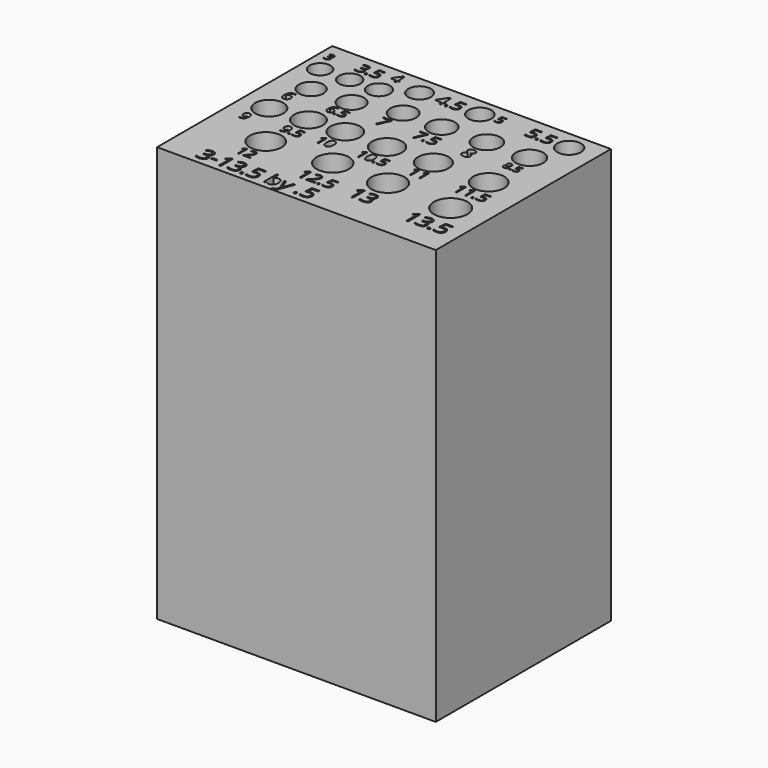
from build123d import *

# Parameters (mm, degrees)
F0_W     = 187.4311566353
F0_H     = 147.2392380238
F0_W_2   = 3.4956519359
F0_H_2   = 1.0824215577
F0_R     = 10.7
F0_R_2   = 9.5
F0_R_3   = 10.9
F0_R_4   = 11.1
F0_R_5   = 11.3
F0_R_6   = 9.7
F0_R_7   = 8.225
F0_R_8   = 9.9
F0_R_9   = 8.45
F0_R_10  = 7
F0_R_11  = 7.2
F0_R_12  = 7.4
F0_R_13  = 8.65
F0_R_14  = 7.6
F0_R_15  = 10.1
F0_R_16  = 10.3
F0_R_17  = 10.5
F0_R_18  = 8.85
F0_R_19  = 9.1
F0_R_20  = 7.8
F0_R_21  = 9.3
F0_R_22  = 8
F1_DEPTH = 279.4


with BuildPart() as f1:
    # F0 (on Top) → F1 (new body)
    with BuildSketch(Plane.XY):
        with Locations((17.0075669885, 2.1902993321)):
            Rectangle(F0_W, F0_H)
        with Locations((-44.6667059077, -63.4352376659)):
            Rectangle(F0_W_2, F0_H_2, mode=Mode.SUBTRACT)
        with BuildLine():
            add(Edge.make_bspline(
                [(-49.0282950899, -57.478500925), (-48.1874244482, -58.1723901131), (-48.1874244482, -59.3824234756)],
                knots=[0, 0, 0, 1, 1, 1], degree=2))
            add(Edge.make_bspline(
                [(-48.1874244482, -59.3824234756), (-48.1874244482, -60.3805300909), (-48.7468654848, -61.01403155)],
                knots=[0, 0, 0, 1, 1, 1], degree=2))
            add(Edge.make_bspline(
                [(-48.7468654848, -61.01403155), (-49.3063065215, -61.647533009), (-50.3317585236, -61.8617385383)],
                knots=[0, 0, 0, 1, 1, 1], degree=2))
            Line((-50.3317585236, -61.8617385383), (-50.3317585236, -61.918708094))
            add(Edge.make_bspline(
                [(-50.3317585236, -61.918708094), (-49.0784282988, -62.0736652854), (-48.4734116176, -62.7151424823)],
                knots=[0, 0, 0, 1, 1, 1], degree=2))
            add(Edge.make_bspline(
                [(-48.4734116176, -62.7151424823), (-47.8683949364, -63.3566196791), (-47.8683949364, -64.3957443746)],
                knots=[0, 0, 0, 1, 1, 1], degree=2))
            add(Edge.make_bspline(
                [(-47.8683949364, -64.3957443746), (-47.8683949364, -65.8837891687), (-48.9006832852, -66.6859205125)],
                knots=[0, 0, 0, 1, 1, 1], degree=2))
            add(Edge.make_bspline(
                [(-48.9006832852, -66.6859205125), (-49.9329716339, -67.4880518563), (-51.8334760111, -67.4880518563)],
                knots=[0, 0, 0, 1, 1, 1], degree=2))
            add(Edge.make_bspline(
                [(-51.8334760111, -67.4880518563), (-52.6606739594, -67.4880518563), (-53.3477268008, -67.3627188339)],
                knots=[0, 0, 0, 1, 1, 1], degree=2))
            add(Edge.make_bspline(
                [(-53.3477268008, -67.3627188339), (-54.0347796422, -67.2373858114), (-54.6819537946, -66.9251926463)],
                knots=[0, 0, 0, 1, 1, 1], degree=2))
            Line((-54.6819537946, -66.9251926463), (-54.6819537946, -65.7994742263))
            add(Edge.make_bspline(
                [(-54.6819537946, -65.7994742263), (-54.0051554732, -66.1344552136), (-53.239484645, -66.308782054)],
                knots=[0, 0, 0, 1, 1, 1], degree=2))
            add(Edge.make_bspline(
                [(-53.239484645, -66.308782054), (-52.4738138168, -66.4831088943), (-51.7901791488, -66.4831088943)],
                knots=[0, 0, 0, 1, 1, 1], degree=2))
            add(Edge.make_bspline(
                [(-51.7901791488, -66.4831088943), (-49.0921009922, -66.4831088943), (-49.0921009922, -64.3683989878)],
                knots=[0, 0, 0, 1, 1, 1], degree=2))
            add(Edge.make_bspline(
                [(-49.0921009922, -64.3683989878), (-49.0921009922, -62.4724521751), (-52.0681905804, -62.4724521751)],
                knots=[0, 0, 0, 1, 1, 1], degree=2))
            Line((-52.0681905804, -62.4724521751), (-53.0936425825, -62.4724521751))
            Line((-53.0936425825, -62.4724521751), (-53.0936425825, -61.456115302))
            Line((-53.0936425825, -61.456115302), (-52.0545178871, -61.456115302))
            add(Edge.make_bspline(
                [(-52.0545178871, -61.456115302), (-50.837648178, -61.456115302), (-50.1255287321, -60.9183226964)],
                knots=[0, 0, 0, 1, 1, 1], degree=2))
            add(Edge.make_bspline(
                [(-50.1255287321, -60.9183226964), (-49.4134092862, -60.3805300909), (-49.4134092862, -59.4257203379)],
                knots=[0, 0, 0, 1, 1, 1], degree=2))
            add(Edge.make_bspline(
                [(-49.4134092862, -59.4257203379), (-49.4134092862, -58.6646070741), (-49.9363898072, -58.2293596688)],
                knots=[0, 0, 0, 1, 1, 1], degree=2))
            add(Edge.make_bspline(
                [(-49.9363898072, -58.2293596688), (-50.4593703283, -57.7941122635), (-51.3572105257, -57.7941122635)],
                knots=[0, 0, 0, 1, 1, 1], degree=2))
            add(Edge.make_bspline(
                [(-51.3572105257, -57.7941122635), (-52.0408451937, -57.7941122635), (-52.6458618749, -57.9798330149)],
                knots=[0, 0, 0, 1, 1, 1], degree=2))
            add(Edge.make_bspline(
                [(-52.6458618749, -57.9798330149), (-53.2508785562, -58.1655537664), (-54.0279432955, -58.6646070741)],
                knots=[0, 0, 0, 1, 1, 1], degree=2))
            Line((-54.0279432955, -58.6646070741), (-54.6249842389, -57.8670332947))
            add(Edge.make_bspline(
                [(-54.6249842389, -57.8670332947), (-53.9846464332, -57.3611436404), (-53.1483333559, -57.0728776887)],
                knots=[0, 0, 0, 1, 1, 1], degree=2))
            add(Edge.make_bspline(
                [(-53.1483333559, -57.0728776887), (-52.3120202787, -56.784611737), (-51.3845559124, -56.784611737)],
                knots=[0, 0, 0, 1, 1, 1], degree=2))
            add(Edge.make_bspline(
                [(-51.3845559124, -56.784611737), (-49.8691657316, -56.784611737), (-49.0282950899, -57.478500925)],
                knots=[0, 0, 0, 1, 1, 1], degree=2))
        make_face(mode=Mode.SUBTRACT)
        with BuildLine():
            Line((-37.2310395016, -56.9327325817), (-37.2310395016, -67.3444885761))
            Line((-37.2310395016, -67.3444885761), (-38.3841033084, -67.3444885761))
            Line((-38.3841033084, -67.3444885761), (-38.3841033084, -59.9247736455))
            add(Edge.make_bspline(
                [(-38.3841033084, -59.9247736455), (-38.3841033084, -58.9973092792), (-38.3271337527, -58.1723901131)],
                knots=[0, 0, 0, 1, 1, 1], degree=2))
            add(Edge.make_bspline(
                [(-38.3271337527, -58.1723901131), (-38.4752545975, -58.3227897401), (-38.660975349, -58.4857226693)],
                knots=[0, 0, 0, 1, 1, 1], degree=2))
            add(Edge.make_bspline(
                [(-38.660975349, -58.4857226693), (-38.8466961004, -58.6486555985), (-40.3552499346, -59.8746404365)],
                knots=[0, 0, 0, 1, 1, 1], degree=2))
            Line((-40.3552499346, -59.8746404365), (-40.981915047, -59.0633939638))
            Line((-40.981915047, -59.0633939638), (-38.2268673347, -56.9327325817))
            Line((-38.2268673347, -56.9327325817), (-37.2310395016, -56.9327325817))
        make_face(mode=Mode.SUBTRACT)
        with BuildLine():
            add(Edge.make_bspline(
                [(-27.660154149, -57.478500925), (-26.8192835073, -58.1723901131), (-26.8192835073, -59.3824234756)],
                knots=[0, 0, 0, 1, 1, 1], degree=2))
            add(Edge.make_bspline(
                [(-26.8192835073, -59.3824234756), (-26.8192835073, -60.3805300909), (-27.378724544, -61.01403155)],
                knots=[0, 0, 0, 1, 1, 1], degree=2))
            add(Edge.make_bspline(
                [(-27.378724544, -61.01403155), (-27.9381655807, -61.647533009), (-28.9636175827, -61.8617385383)],
                knots=[0, 0, 0, 1, 1, 1], degree=2))
            Line((-28.9636175827, -61.8617385383), (-28.9636175827, -61.918708094))
            add(Edge.make_bspline(
                [(-28.9636175827, -61.918708094), (-27.710287358, -62.0736652854), (-27.1052706768, -62.7151424823)],
                knots=[0, 0, 0, 1, 1, 1], degree=2))
            add(Edge.make_bspline(
                [(-27.1052706768, -62.7151424823), (-26.5002539955, -63.3566196791), (-26.5002539955, -64.3957443746)],
                knots=[0, 0, 0, 1, 1, 1], degree=2))
            add(Edge.make_bspline(
                [(-26.5002539955, -64.3957443746), (-26.5002539955, -65.8837891687), (-27.5325423443, -66.6859205125)],
                knots=[0, 0, 0, 1, 1, 1], degree=2))
            add(Edge.make_bspline(
                [(-27.5325423443, -66.6859205125), (-28.564830693, -67.4880518563), (-30.4653350702, -67.4880518563)],
                knots=[0, 0, 0, 1, 1, 1], degree=2))
            add(Edge.make_bspline(
                [(-30.4653350702, -67.4880518563), (-31.2925330185, -67.4880518563), (-31.9795858599, -67.3627188339)],
                knots=[0, 0, 0, 1, 1, 1], degree=2))
            add(Edge.make_bspline(
                [(-31.9795858599, -67.3627188339), (-32.6666387013, -67.2373858114), (-33.3138128537, -66.9251926463)],
                knots=[0, 0, 0, 1, 1, 1], degree=2))
            Line((-33.3138128537, -66.9251926463), (-33.3138128537, -65.7994742263))
            add(Edge.make_bspline(
                [(-33.3138128537, -65.7994742263), (-32.6370145324, -66.1344552136), (-31.8713437041, -66.308782054)],
                knots=[0, 0, 0, 1, 1, 1], degree=2))
            add(Edge.make_bspline(
                [(-31.8713437041, -66.308782054), (-31.1056728759, -66.4831088943), (-30.4220382079, -66.4831088943)],
                knots=[0, 0, 0, 1, 1, 1], degree=2))
            add(Edge.make_bspline(
                [(-30.4220382079, -66.4831088943), (-27.7239600513, -66.4831088943), (-27.7239600513, -64.3683989878)],
                knots=[0, 0, 0, 1, 1, 1], degree=2))
            add(Edge.make_bspline(
                [(-27.7239600513, -64.3683989878), (-27.7239600513, -62.4724521751), (-30.7000496396, -62.4724521751)],
                knots=[0, 0, 0, 1, 1, 1], degree=2))
            Line((-30.7000496396, -62.4724521751), (-31.7255016416, -62.4724521751))
            Line((-31.7255016416, -62.4724521751), (-31.7255016416, -61.456115302))
            Line((-31.7255016416, -61.456115302), (-30.6863769462, -61.456115302))
            add(Edge.make_bspline(
                [(-30.6863769462, -61.456115302), (-29.4695072371, -61.456115302), (-28.7573877912, -60.9183226964)],
                knots=[0, 0, 0, 1, 1, 1], degree=2))
            add(Edge.make_bspline(
                [(-28.7573877912, -60.9183226964), (-28.0452683453, -60.3805300909), (-28.0452683453, -59.4257203379)],
                knots=[0, 0, 0, 1, 1, 1], degree=2))
            add(Edge.make_bspline(
                [(-28.0452683453, -59.4257203379), (-28.0452683453, -58.6646070741), (-28.5682488664, -58.2293596688)],
                knots=[0, 0, 0, 1, 1, 1], degree=2))
            add(Edge.make_bspline(
                [(-28.5682488664, -58.2293596688), (-29.0912293874, -57.7941122635), (-29.9890695848, -57.7941122635)],
                knots=[0, 0, 0, 1, 1, 1], degree=2))
            add(Edge.make_bspline(
                [(-29.9890695848, -57.7941122635), (-30.6727042528, -57.7941122635), (-31.2777209341, -57.9798330149)],
                knots=[0, 0, 0, 1, 1, 1], degree=2))
            add(Edge.make_bspline(
                [(-31.2777209341, -57.9798330149), (-31.8827376153, -58.1655537664), (-32.6598023546, -58.6646070741)],
                knots=[0, 0, 0, 1, 1, 1], degree=2))
            Line((-32.6598023546, -58.6646070741), (-33.2568432981, -57.8670332947))
            add(Edge.make_bspline(
                [(-33.2568432981, -57.8670332947), (-32.6165054923, -57.3611436404), (-31.7801924151, -57.0728776887)],
                knots=[0, 0, 0, 1, 1, 1], degree=2))
            add(Edge.make_bspline(
                [(-31.7801924151, -57.0728776887), (-30.9438793378, -56.784611737), (-30.0164149715, -56.784611737)],
                knots=[0, 0, 0, 1, 1, 1], degree=2))
            add(Edge.make_bspline(
                [(-30.0164149715, -56.784611737), (-28.5010247907, -56.784611737), (-27.660154149, -57.478500925)],
                knots=[0, 0, 0, 1, 1, 1], degree=2))
        make_face(mode=Mode.SUBTRACT)
        with BuildLine():
            Line((-38.3842547211, -43.3635103836), (-38.3842547211, -50.5557730794))
            Line((-38.3842547211, -50.5557730794), (-39.1807714477, -50.5557730794))
            Line((-39.1807714477, -50.5557730794), (-39.1807714477, -45.4303610992))
            add(Edge.make_bspline(
                [(-39.1807714477, -45.4303610992), (-39.1807714477, -44.7896846017), (-39.1414178545, -44.219844572)],
                knots=[0, 0, 0, 1, 1, 1], degree=2))
            add(Edge.make_bspline(
                [(-39.1414178545, -44.219844572), (-39.2437371969, -44.3237380581), (-39.3720299107, -44.4362893347)],
                knots=[0, 0, 0, 1, 1, 1], degree=2))
            add(Edge.make_bspline(
                [(-39.3720299107, -44.4362893347), (-39.5003226246, -44.5488406112), (-40.5424057729, -45.3957299372)],
                knots=[0, 0, 0, 1, 1, 1], degree=2))
            Line((-40.5424057729, -45.3957299372), (-40.9752952983, -44.8353347698))
            Line((-40.9752952983, -44.8353347698), (-39.0721555304, -43.3635103836))
            Line((-39.0721555304, -43.3635103836), (-38.3842547211, -43.3635103836))
        make_face(mode=Mode.SUBTRACT)
        with BuildLine():
            Line((-30.921239304, -49.798609946), (-30.921239304, -50.5557730794))
            Line((-30.921239304, -50.5557730794), (-35.6483929208, -50.5557730794))
            Line((-35.6483929208, -50.5557730794), (-35.6483929208, -49.8521308327))
            Line((-35.6483929208, -49.8521308327), (-33.7546980154, -47.9489910649))
            add(Edge.make_bspline(
                [(-33.7546980154, -47.9489910649), (-32.8889189647, -47.0721930081), (-32.6134438122, -46.6983338726)],
                knots=[0, 0, 0, 1, 1, 1], degree=2))
            add(Edge.make_bspline(
                [(-32.6134438122, -46.6983338726), (-32.3379686597, -46.324474737), (-32.2002310835, -45.9702923981)],
                knots=[0, 0, 0, 1, 1, 1], degree=2))
            add(Edge.make_bspline(
                [(-32.2002310835, -45.9702923981), (-32.0624935072, -45.6161100592), (-32.0624935072, -45.2084068335)],
                knots=[0, 0, 0, 1, 1, 1], degree=2))
            add(Edge.make_bspline(
                [(-32.0624935072, -45.2084068335), (-32.0624935072, -44.6322702289), (-32.4119534149, -44.2954034709)],
                knots=[0, 0, 0, 1, 1, 1], degree=2))
            add(Edge.make_bspline(
                [(-32.4119534149, -44.2954034709), (-32.7614133227, -43.958536713), (-33.3816259517, -43.958536713)],
                knots=[0, 0, 0, 1, 1, 1], degree=2))
            add(Edge.make_bspline(
                [(-33.3816259517, -43.958536713), (-33.8286827706, -43.958536713), (-34.2300894214, -44.1065062235)],
                knots=[0, 0, 0, 1, 1, 1], degree=2))
            add(Edge.make_bspline(
                [(-34.2300894214, -44.1065062235), (-34.6314960722, -44.254475734), (-35.1226289155, -44.643289235)],
                knots=[0, 0, 0, 1, 1, 1], degree=2))
            Line((-35.1226289155, -44.643289235), (-35.5555184409, -44.0876164988))
            add(Edge.make_bspline(
                [(-35.5555184409, -44.0876164988), (-34.5622337481, -43.2611910413), (-33.3910708141, -43.2611910413)],
                knots=[0, 0, 0, 1, 1, 1], degree=2))
            add(Edge.make_bspline(
                [(-33.3910708141, -43.2611910413), (-32.3773222529, -43.2611910413), (-31.8019727201, -43.7798713998)],
                knots=[0, 0, 0, 1, 1, 1], degree=2))
            add(Edge.make_bspline(
                [(-31.8019727201, -43.7798713998), (-31.2266231873, -44.2985517584), (-31.2266231873, -45.1737756715)],
                knots=[0, 0, 0, 1, 1, 1], degree=2))
            add(Edge.make_bspline(
                [(-31.2266231873, -45.1737756715), (-31.2266231873, -45.8585281934), (-31.6107142571, -46.527539278)],
                knots=[0, 0, 0, 1, 1, 1], degree=2))
            add(Edge.make_bspline(
                [(-31.6107142571, -46.527539278), (-31.9948053269, -47.1965503627), (-33.0463333376, -48.2197437862)],
                knots=[0, 0, 0, 1, 1, 1], degree=2))
            Line((-33.0463333376, -48.2197437862), (-34.6204770661, -49.7592563527))
            Line((-34.6204770661, -49.7592563527), (-34.6204770661, -49.798609946))
            Line((-34.6204770661, -49.798609946), (-30.921239304, -49.798609946))
        make_face(mode=Mode.SUBTRACT)
        with BuildLine():
            add(Edge.make_bspline(
                [(-24.32515636, -67.3273977094), (-24.5632891027, -67.10293766), (-24.5632891027, -66.590211659)],
                knots=[0, 0, 0, 1, 1, 1], degree=2))
            add(Edge.make_bspline(
                [(-24.5632891027, -66.590211659), (-24.5632891027, -66.1116673913), (-24.3456654001, -65.866698302)],
                knots=[0, 0, 0, 1, 1, 1], degree=2))
            add(Edge.make_bspline(
                [(-24.3456654001, -65.866698302), (-24.1280416974, -65.6217292126), (-23.722418461, -65.6217292126)],
                knots=[0, 0, 0, 1, 1, 1], degree=2))
            add(Edge.make_bspline(
                [(-23.722418461, -65.6217292126), (-23.309958878, -65.6217292126), (-23.078662482, -65.866698302)],
                knots=[0, 0, 0, 1, 1, 1], degree=2))
            add(Edge.make_bspline(
                [(-23.078662482, -65.866698302), (-22.8473660859, -66.1116673913), (-22.8473660859, -66.590211659)],
                knots=[0, 0, 0, 1, 1, 1], degree=2))
            add(Edge.make_bspline(
                [(-22.8473660859, -66.590211659), (-22.8473660859, -67.052804451), (-23.0820806553, -67.3023311049)],
                knots=[0, 0, 0, 1, 1, 1], degree=2))
            add(Edge.make_bspline(
                [(-23.0820806553, -67.3023311049), (-23.3167952247, -67.5518577587), (-23.722418461, -67.5518577587)],
                knots=[0, 0, 0, 1, 1, 1], degree=2))
            add(Edge.make_bspline(
                [(-23.722418461, -67.5518577587), (-24.0870236173, -67.5518577587), (-24.32515636, -67.3273977094)],
                knots=[0, 0, 0, 1, 1, 1], degree=2))
        make_face(mode=Mode.SUBTRACT)
        with BuildLine():
            add(Edge.make_bspline(
                [(-19.4291927457, -61.1484797013), (-18.6111099263, -60.984407381), (-17.7975846713, -60.984407381)],
                knots=[0, 0, 0, 1, 1, 1], degree=2))
            add(Edge.make_bspline(
                [(-17.7975846713, -60.984407381), (-16.1523039036, -60.984407381), (-15.2088880617, -61.8002114182)],
                knots=[0, 0, 0, 1, 1, 1], degree=2))
            add(Edge.make_bspline(
                [(-15.2088880617, -61.8002114182), (-14.2654722198, -62.6160154554), (-14.2654722198, -64.0334180005)],
                knots=[0, 0, 0, 1, 1, 1], degree=2))
            add(Edge.make_bspline(
                [(-14.2654722198, -64.0334180005), (-14.2654722198, -65.6490745993), (-15.2943423952, -66.5685632278)],
                knots=[0, 0, 0, 1, 1, 1], degree=2))
            add(Edge.make_bspline(
                [(-15.2943423952, -66.5685632278), (-16.3232125706, -67.4880518563), (-18.1325656587, -67.4880518563)],
                knots=[0, 0, 0, 1, 1, 1], degree=2))
            add(Edge.make_bspline(
                [(-18.1325656587, -67.4880518563), (-19.8917855378, -67.4880518563), (-20.8169711219, -66.9251926463)],
                knots=[0, 0, 0, 1, 1, 1], degree=2))
            Line((-20.8169711219, -66.9251926463), (-20.8169711219, -65.7858015329))
            add(Edge.make_bspline(
                [(-20.8169711219, -65.7858015329), (-20.3201965964, -66.1048310447), (-19.5795923727, -66.2871336228)],
                knots=[0, 0, 0, 1, 1, 1], degree=2))
            add(Edge.make_bspline(
                [(-19.5795923727, -66.2871336228), (-18.838988149, -66.469436201), (-18.1188929653, -66.469436201)],
                knots=[0, 0, 0, 1, 1, 1], degree=2))
            add(Edge.make_bspline(
                [(-18.1188929653, -66.469436201), (-16.8655627406, -66.469436201), (-16.1716735525, -65.8780922131)],
                knots=[0, 0, 0, 1, 1, 1], degree=2))
            add(Edge.make_bspline(
                [(-16.1716735525, -65.8780922131), (-15.4777843644, -65.2867482252), (-15.4777843644, -64.1678661519)],
                knots=[0, 0, 0, 1, 1, 1], degree=2))
            add(Edge.make_bspline(
                [(-15.4777843644, -64.1678661519), (-15.4777843644, -61.989350343), (-18.146238352, -61.989350343)],
                knots=[0, 0, 0, 1, 1, 1], degree=2))
            add(Edge.make_bspline(
                [(-18.146238352, -61.989350343), (-18.8230366734, -61.989350343), (-19.9555914401, -62.1967195257)],
                knots=[0, 0, 0, 1, 1, 1], degree=2))
            Line((-19.9555914401, -62.1967195257), (-20.5685838591, -61.8047689827))
            Line((-20.5685838591, -61.8047689827), (-20.1766333161, -56.9327325817))
            Line((-20.1766333161, -56.9327325817), (-14.9992400968, -56.9327325817))
            Line((-14.9992400968, -56.9327325817), (-14.9992400968, -58.0219904861))
            Line((-14.9992400968, -58.0219904861), (-19.1648540074, -58.0219904861))
            Line((-19.1648540074, -58.0219904861), (-19.4291927457, -61.1484797013))
        make_face(mode=Mode.SUBTRACT)
        with BuildLine():
            Line((2.4630681073, -67.3877854384), (-0.6862089301, -59.5396594492))
            Line((-0.6862089301, -59.5396594492), (0.5830727702, -59.5396594492))
            Line((0.5830727702, -59.5396594492), (2.2921594403, -63.9901211382))
            add(Edge.make_bspline(
                [(2.2921594403, -63.9901211382), (2.8527398681, -65.5146264479), (2.9894668017, -66.1914247693)],
                knots=[0, 0, 0, 1, 1, 1], degree=2))
            Line((2.9894668017, -66.1914247693), (3.0464363574, -66.1914247693))
            add(Edge.make_bspline(
                [(3.0464363574, -66.1914247693), (3.1375876465, -65.826819613), (3.4338293359, -64.9472096734)],
                knots=[0, 0, 0, 1, 1, 1], degree=2))
            add(Edge.make_bspline(
                [(3.4338293359, -64.9472096734), (3.7300710254, -64.0675997339), (5.3685154465, -59.5396594492)],
                knots=[0, 0, 0, 1, 1, 1], degree=2))
            Line((5.3685154465, -59.5396594492), (6.6355183646, -59.5396594492))
            Line((6.6355183646, -59.5396594492), (3.2811509267, -68.4269101338))
            add(Edge.make_bspline(
                [(3.2811509267, -68.4269101338), (2.7820976191, -69.7440462609), (2.1166932088, -70.2966509509)],
                knots=[0, 0, 0, 1, 1, 1], degree=2))
            add(Edge.make_bspline(
                [(2.1166932088, -70.2966509509), (1.4512887986, -70.8492556409), (0.4828063522, -70.8492556409)],
                knots=[0, 0, 0, 1, 1, 1], degree=2))
            add(Edge.make_bspline(
                [(0.4828063522, -70.8492556409), (-0.0595438178, -70.8492556409), (-0.5859425122, -70.7262014007)],
                knots=[0, 0, 0, 1, 1, 1], degree=2))
            Line((-0.5859425122, -70.7262014007), (-0.5859425122, -69.7805067765))
            add(Edge.make_bspline(
                [(-0.5859425122, -69.7805067765), (-0.1939919692, -69.8648217189), (0.2891098629, -69.8648217189)],
                knots=[0, 0, 0, 1, 1, 1], degree=2))
            add(Edge.make_bspline(
                [(0.2891098629, -69.8648217189), (1.5082583543, -69.8648217189), (2.027820702, -68.4975523828)],
                knots=[0, 0, 0, 1, 1, 1], degree=2))
            Line((2.027820702, -68.4975523828), (2.4630681073, -67.3877854384))
        make_face(mode=Mode.SUBTRACT)
        with BuildLine():
            add(Edge.make_bspline(
                [(11.7593602016, -67.3273977094), (11.5212274589, -67.10293766), (11.5212274589, -66.590211659)],
                knots=[0, 0, 0, 1, 1, 1], degree=2))
            add(Edge.make_bspline(
                [(11.5212274589, -66.590211659), (11.5212274589, -66.1116673913), (11.7388511616, -65.866698302)],
                knots=[0, 0, 0, 1, 1, 1], degree=2))
            add(Edge.make_bspline(
                [(11.7388511616, -65.866698302), (11.9564748642, -65.6217292126), (12.3620981006, -65.6217292126)],
                knots=[0, 0, 0, 1, 1, 1], degree=2))
            add(Edge.make_bspline(
                [(12.3620981006, -65.6217292126), (12.7745576837, -65.6217292126), (13.0058540797, -65.866698302)],
                knots=[0, 0, 0, 1, 1, 1], degree=2))
            add(Edge.make_bspline(
                [(13.0058540797, -65.866698302), (13.2371504757, -66.1116673913), (13.2371504757, -66.590211659)],
                knots=[0, 0, 0, 1, 1, 1], degree=2))
            add(Edge.make_bspline(
                [(13.2371504757, -66.590211659), (13.2371504757, -67.052804451), (13.0024359064, -67.3023311049)],
                knots=[0, 0, 0, 1, 1, 1], degree=2))
            add(Edge.make_bspline(
                [(13.0024359064, -67.3023311049), (12.767721337, -67.5518577587), (12.3620981006, -67.5518577587)],
                knots=[0, 0, 0, 1, 1, 1], degree=2))
            add(Edge.make_bspline(
                [(12.3620981006, -67.5518577587), (11.9974929443, -67.5518577587), (11.7593602016, -67.3273977094)],
                knots=[0, 0, 0, 1, 1, 1], degree=2))
        make_face(mode=Mode.SUBTRACT)
        with BuildLine():
            add(Edge.make_bspline(
                [(-7.2012473166, -60.5787841446), (-6.3763281505, -59.4120476445), (-4.7515564228, -59.4120476445)],
                knots=[0, 0, 0, 1, 1, 1], degree=2))
            add(Edge.make_bspline(
                [(-4.7515564228, -59.4120476445), (-3.2133784197, -59.4120476445), (-2.362253258, -60.4625662511)],
                knots=[0, 0, 0, 1, 1, 1], degree=2))
            add(Edge.make_bspline(
                [(-2.362253258, -60.4625662511), (-1.5111280963, -61.5130848576), (-1.5111280963, -63.4340982748)],
                knots=[0, 0, 0, 1, 1, 1], degree=2))
            add(Edge.make_bspline(
                [(-1.5111280963, -63.4340982748), (-1.5111280963, -65.3573904743), (-2.3690896046, -66.4227211653)],
                knots=[0, 0, 0, 1, 1, 1], degree=2))
            add(Edge.make_bspline(
                [(-2.3690896046, -66.4227211653), (-3.227051113, -67.4880518563), (-4.7515564228, -67.4880518563)],
                knots=[0, 0, 0, 1, 1, 1], degree=2))
            add(Edge.make_bspline(
                [(-4.7515564228, -67.4880518563), (-5.5149484688, -67.4880518563), (-6.1450317545, -67.2066222513)],
                knots=[0, 0, 0, 1, 1, 1], degree=2))
            add(Edge.make_bspline(
                [(-6.1450317545, -67.2066222513), (-6.7751150402, -66.9251926463), (-7.2012473166, -66.339545614)],
                knots=[0, 0, 0, 1, 1, 1], degree=2))
            Line((-7.2012473166, -66.339545614), (-7.2878410412, -66.339545614))
            Line((-7.2878410412, -66.339545614), (-7.536228304, -67.3444885761))
            Line((-7.536228304, -67.3444885761), (-8.3839352923, -67.3444885761))
            Line((-8.3839352923, -67.3444885761), (-8.3839352923, -56.262770607))
            Line((-8.3839352923, -56.262770607), (-7.2012473166, -56.262770607))
            Line((-7.2012473166, -56.262770607), (-7.2012473166, -58.9562911991))
            add(Edge.make_bspline(
                [(-7.2012473166, -58.9562911991), (-7.2012473166, -59.8609677432), (-7.2582168723, -60.5787841446)],
                knots=[0, 0, 0, 1, 1, 1], degree=2))
            Line((-7.2582168723, -60.5787841446), (-7.2012473166, -60.5787841446))
        make_face(mode=Mode.SUBTRACT)
        with BuildLine():
            Line((4.2081283496, -42.9125359418), (4.2081283496, -51.5190437436))
            Line((4.2081283496, -51.5190437436), (3.2549891621, -51.5190437436))
            Line((3.2549891621, -51.5190437436), (3.2549891621, -45.3858002762))
            add(Edge.make_bspline(
                [(3.2549891621, -45.3858002762), (3.2549891621, -44.6191448427), (3.3020810192, -43.9372547521)],
                knots=[0, 0, 0, 1, 1, 1], degree=2))
            add(Edge.make_bspline(
                [(3.3020810192, -43.9372547521), (3.1796421907, -44.0615772548), (3.0261227366, -44.1962599661)],
                knots=[0, 0, 0, 1, 1, 1], degree=2))
            add(Edge.make_bspline(
                [(3.0261227366, -44.1962599661), (2.8726032825, -44.3309426773), (1.6256109068, -45.3443594419)],
                knots=[0, 0, 0, 1, 1, 1], degree=2))
            Line((1.6256109068, -45.3443594419), (1.1076004788, -44.673771397))
            Line((1.1076004788, -44.673771397), (3.3849626877, -42.9125359418))
            Line((3.3849626877, -42.9125359418), (4.2081283496, -42.9125359418))
        make_face(mode=Mode.SUBTRACT)
        with BuildLine():
            add(Edge.make_bspline(
                [(14.8763176549, -51.5049161865), (14.6794736922, -51.3193742695), (14.6794736922, -50.8955475557)],
                knots=[0, 0, 0, 1, 1, 1], degree=2))
            add(Edge.make_bspline(
                [(14.6794736922, -50.8955475557), (14.6794736922, -50.4999759562), (14.8593645863, -50.2974809707)],
                knots=[0, 0, 0, 1, 1, 1], degree=2))
            add(Edge.make_bspline(
                [(14.8593645863, -50.2974809707), (15.0392554804, -50.0949859852), (15.3745495029, -50.0949859852)],
                knots=[0, 0, 0, 1, 1, 1], degree=2))
            add(Edge.make_bspline(
                [(15.3745495029, -50.0949859852), (15.7154945482, -50.0949859852), (15.906687488, -50.2974809707)],
                knots=[0, 0, 0, 1, 1, 1], degree=2))
            add(Edge.make_bspline(
                [(15.906687488, -50.2974809707), (16.0978804278, -50.4999759562), (16.0978804278, -50.8955475557)],
                knots=[0, 0, 0, 1, 1, 1], degree=2))
            add(Edge.make_bspline(
                [(16.0978804278, -50.8955475557), (16.0978804278, -51.2779334353), (15.9038619766, -51.4841957694)],
                knots=[0, 0, 0, 1, 1, 1], degree=2))
            add(Edge.make_bspline(
                [(15.9038619766, -51.4841957694), (15.7098435254, -51.6904581034), (15.3745495029, -51.6904581034)],
                knots=[0, 0, 0, 1, 1, 1], degree=2))
            add(Edge.make_bspline(
                [(15.3745495029, -51.6904581034), (15.0731616175, -51.6904581034), (14.8763176549, -51.5049161865)],
                knots=[0, 0, 0, 1, 1, 1], degree=2))
        make_face(mode=Mode.SUBTRACT)
        with BuildLine():
            Line((13.1386281282, -50.6129964132), (13.1386281282, -51.5190437436))
            Line((13.1386281282, -51.5190437436), (7.4819542545, -51.5190437436))
            Line((7.4819542545, -51.5190437436), (7.4819542545, -50.6770413388))
            Line((7.4819542545, -50.6770413388), (9.7480144177, -48.3996791299))
            add(Edge.make_bspline(
                [(9.7480144177, -48.3996791299), (10.7840352737, -47.350472554), (11.1136782733, -46.9030999116)],
                knots=[0, 0, 0, 1, 1, 1], degree=2))
            add(Edge.make_bspline(
                [(11.1136782733, -46.9030999116), (11.443321273, -46.4557272693), (11.6081427728, -46.0319005554)],
                knots=[0, 0, 0, 1, 1, 1], degree=2))
            add(Edge.make_bspline(
                [(11.6081427728, -46.0319005554), (11.7729642726, -45.6080738416), (11.7729642726, -45.1202022022)],
                knots=[0, 0, 0, 1, 1, 1], degree=2))
            add(Edge.make_bspline(
                [(11.7729642726, -45.1202022022), (11.7729642726, -44.4307774144), (11.3547885816, -44.0276711177)],
                knots=[0, 0, 0, 1, 1, 1], degree=2))
            add(Edge.make_bspline(
                [(11.3547885816, -44.0276711177), (10.9366128907, -43.624564821), (10.1944452229, -43.624564821)],
                knots=[0, 0, 0, 1, 1, 1], degree=2))
            add(Edge.make_bspline(
                [(10.1944452229, -43.624564821), (9.6594817264, -43.624564821), (9.1791447841, -43.8016302036)],
                knots=[0, 0, 0, 1, 1, 1], degree=2))
            add(Edge.make_bspline(
                [(9.1791447841, -43.8016302036), (8.6988078417, -43.9786955863), (8.1111014652, -44.4439631344)],
                knots=[0, 0, 0, 1, 1, 1], degree=2))
            Line((8.1111014652, -44.4439631344), (7.5930910373, -43.7790261122))
            add(Edge.make_bspline(
                [(7.5930910373, -43.7790261122), (8.7816895102, -42.7900971133), (10.1831431772, -42.7900971133)],
                knots=[0, 0, 0, 1, 1, 1], degree=2))
            add(Edge.make_bspline(
                [(10.1831431772, -42.7900971133), (11.3962294159, -42.7900971133), (12.0847123665, -43.4107677898)],
                knots=[0, 0, 0, 1, 1, 1], degree=2))
            add(Edge.make_bspline(
                [(12.0847123665, -43.4107677898), (12.7731953172, -44.0314384662), (12.7731953172, -45.0787613679)],
                knots=[0, 0, 0, 1, 1, 1], degree=2))
            add(Edge.make_bspline(
                [(12.7731953172, -45.0787613679), (12.7731953172, -45.8981596813), (12.313578792, -46.6987212518)],
                knots=[0, 0, 0, 1, 1, 1], degree=2))
            add(Edge.make_bspline(
                [(12.313578792, -46.6987212518), (11.8539622668, -47.4992828224), (10.5956678453, -48.7236711067)],
                knots=[0, 0, 0, 1, 1, 1], degree=2))
            Line((10.5956678453, -48.7236711067), (8.7119935617, -50.5659045561))
            Line((8.7119935617, -50.5659045561), (8.7119935617, -50.6129964132))
            Line((8.7119935617, -50.6129964132), (13.1386281282, -50.6129964132))
        make_face(mode=Mode.SUBTRACT)
        with Locations((-36.1858941615, -30.7730771601)):
            Circle(F0_R, mode=Mode.SUBTRACT)
        with BuildLine():
            add(Edge.make_bspline(
                [(-60.7940741832, -12.5551076529), (-60.5168102896, -13.2316315533), (-60.5168102896, -14.1514083098)],
                knots=[0, 0, 0, 1, 1, 1], degree=2))
            add(Edge.make_bspline(
                [(-60.5168102896, -14.1514083098), (-60.5168102896, -18.1173910441), (-63.585197379, -18.1173910441)],
                knots=[0, 0, 0, 1, 1, 1], degree=2))
            add(Edge.make_bspline(
                [(-63.585197379, -18.1173910441), (-64.1219802771, -18.1173910441), (-64.4354733195, -18.0242303759)],
                knots=[0, 0, 0, 1, 1, 1], degree=2))
            Line((-64.4354733195, -18.0242303759), (-64.4354733195, -17.3632332535))
            add(Edge.make_bspline(
                [(-64.4354733195, -17.3632332535), (-64.065788128, -17.4830112555), (-63.5955485644, -17.4830112555)],
                knots=[0, 0, 0, 1, 1, 1], degree=2))
            add(Edge.make_bspline(
                [(-63.5955485644, -17.4830112555), (-62.4864929899, -17.4830112555), (-61.9201352765, -16.7968755401)],
                knots=[0, 0, 0, 1, 1, 1], degree=2))
            add(Edge.make_bspline(
                [(-61.9201352765, -16.7968755401), (-61.3537775632, -16.1107398247), (-61.3035003771, -14.6926274301)],
                knots=[0, 0, 0, 1, 1, 1], degree=2))
            Line((-61.3035003771, -14.6926274301), (-61.3582137854, -14.6926274301))
            add(Edge.make_bspline(
                [(-61.3582137854, -14.6926274301), (-61.6125571972, -15.0756212885), (-62.0332589451, -15.2767300327)],
                knots=[0, 0, 0, 1, 1, 1], degree=2))
            add(Edge.make_bspline(
                [(-62.0332589451, -15.2767300327), (-62.453960693, -15.4778387769), (-62.9803924057, -15.4778387769)],
                knots=[0, 0, 0, 1, 1, 1], degree=2))
            add(Edge.make_bspline(
                [(-62.9803924057, -15.4778387769), (-63.8765093099, -15.4778387769), (-64.403680393, -14.9417952492)],
                knots=[0, 0, 0, 1, 1, 1], degree=2))
            add(Edge.make_bspline(
                [(-64.403680393, -14.9417952492), (-64.9308514761, -14.4057517215), (-64.9308514761, -13.4445702236)],
                knots=[0, 0, 0, 1, 1, 1], degree=2))
            add(Edge.make_bspline(
                [(-64.9308514761, -13.4445702236), (-64.9308514761, -12.3917067982), (-64.3415732808, -11.7817262323)],
                knots=[0, 0, 0, 1, 1, 1], degree=2))
            add(Edge.make_bspline(
                [(-64.3415732808, -11.7817262323), (-63.7522950856, -11.1717456663), (-62.7911135877, -11.1717456663)],
                knots=[0, 0, 0, 1, 1, 1], degree=2))
            add(Edge.make_bspline(
                [(-62.7911135877, -11.1717456663), (-62.1020203907, -11.1717456663), (-61.5866792338, -11.5251647094)],
                knots=[0, 0, 0, 1, 1, 1], degree=2))
            add(Edge.make_bspline(
                [(-61.5866792338, -11.5251647094), (-61.0713380768, -11.8785837525), (-60.7940741832, -12.5551076529)],
                knots=[0, 0, 0, 1, 1, 1], degree=2))
        make_face(mode=Mode.SUBTRACT)
        with Locations((-58.3864711225, 0)):
            Circle(F0_R_2, mode=Mode.SUBTRACT)
        with BuildLine():
            add(Edge.make_bspline(
                [(-34.4877288534, -10.8400304239), (-34.2015209131, -11.5383777983), (-34.2015209131, -12.4878249389)],
                knots=[0, 0, 0, 1, 1, 1], degree=2))
            add(Edge.make_bspline(
                [(-34.2015209131, -12.4878249389), (-34.2015209131, -16.5817433171), (-37.3688887859, -16.5817433171)],
                knots=[0, 0, 0, 1, 1, 1], degree=2))
            add(Edge.make_bspline(
                [(-37.3688887859, -16.5817433171), (-37.9229873583, -16.5817433171), (-38.2465931361, -16.4855774492)],
                knots=[0, 0, 0, 1, 1, 1], degree=2))
            Line((-38.2465931361, -16.4855774492), (-38.2465931361, -15.8032577195))
            add(Edge.make_bspline(
                [(-38.2465931361, -15.8032577195), (-37.8649825491, -15.9268995497), (-37.3795738823, -15.9268995497)],
                knots=[0, 0, 0, 1, 1, 1], degree=2))
            add(Edge.make_bspline(
                [(-37.3795738823, -15.9268995497), (-36.234742121, -15.9268995497), (-35.6501147016, -15.2186303001)],
                knots=[0, 0, 0, 1, 1, 1], degree=2))
            add(Edge.make_bspline(
                [(-35.6501147016, -15.2186303001), (-35.0654872822, -14.5103610505), (-35.0135882424, -13.0465028384)],
                knots=[0, 0, 0, 1, 1, 1], degree=2))
            Line((-35.0135882424, -13.0465028384), (-35.0700666093, -13.0465028384))
            add(Edge.make_bspline(
                [(-35.0700666093, -13.0465028384), (-35.3326146932, -13.4418514066), (-35.7668875413, -13.649447566)],
                knots=[0, 0, 0, 1, 1, 1], degree=2))
            add(Edge.make_bspline(
                [(-35.7668875413, -13.649447566), (-36.2011603894, -13.8570437254), (-36.7445738654, -13.8570437254)],
                knots=[0, 0, 0, 1, 1, 1], degree=2))
            add(Edge.make_bspline(
                [(-36.7445738654, -13.8570437254), (-37.6695979285, -13.8570437254), (-38.2137746256, -13.3037083741)],
                knots=[0, 0, 0, 1, 1, 1], degree=2))
            add(Edge.make_bspline(
                [(-38.2137746256, -13.3037083741), (-38.7579513228, -12.7503730229), (-38.7579513228, -11.7581854964)],
                knots=[0, 0, 0, 1, 1, 1], degree=2))
            add(Edge.make_bspline(
                [(-38.7579513228, -11.7581854964), (-38.7579513228, -10.6713585444), (-38.149664047, -10.0417010758)],
                knots=[0, 0, 0, 1, 1, 1], degree=2))
            add(Edge.make_bspline(
                [(-38.149664047, -10.0417010758), (-37.5413767712, -9.4120436071), (-36.5491892448, -9.4120436071)],
                knots=[0, 0, 0, 1, 1, 1], degree=2))
            add(Edge.make_bspline(
                [(-36.5491892448, -9.4120436071), (-35.8378671105, -9.4120436071), (-35.3059019521, -9.7768633283)],
                knots=[0, 0, 0, 1, 1, 1], degree=2))
            add(Edge.make_bspline(
                [(-35.3059019521, -9.7768633283), (-34.7739367937, -10.1416830496), (-34.4877288534, -10.8400304239)],
                knots=[0, 0, 0, 1, 1, 1], degree=2))
        make_face(mode=Mode.SUBTRACT)
        with BuildLine():
            add(Edge.make_bspline(
                [(-32.7933778468, -16.4741291316), (-32.9528910722, -16.3237745603), (-32.9528910722, -15.9803250319)],
                knots=[0, 0, 0, 1, 1, 1], degree=2))
            add(Edge.make_bspline(
                [(-32.9528910722, -15.9803250319), (-32.9528910722, -15.6597721388), (-32.8071158279, -15.4956795863)],
                knots=[0, 0, 0, 1, 1, 1], degree=2))
            add(Edge.make_bspline(
                [(-32.8071158279, -15.4956795863), (-32.6613405836, -15.3315870339), (-32.3896338456, -15.3315870339)],
                knots=[0, 0, 0, 1, 1, 1], degree=2))
            add(Edge.make_bspline(
                [(-32.3896338456, -15.3315870339), (-32.1133477806, -15.3315870339), (-31.9584138822, -15.4956795863)],
                knots=[0, 0, 0, 1, 1, 1], degree=2))
            add(Edge.make_bspline(
                [(-31.9584138822, -15.4956795863), (-31.8034799839, -15.6597721388), (-31.8034799839, -15.9803250319)],
                knots=[0, 0, 0, 1, 1, 1], degree=2))
            add(Edge.make_bspline(
                [(-31.8034799839, -15.9803250319), (-31.8034799839, -16.2901928286), (-31.9607035457, -16.4573382658)],
                knots=[0, 0, 0, 1, 1, 1], degree=2))
            add(Edge.make_bspline(
                [(-31.9607035457, -16.4573382658), (-32.1179271076, -16.6244837029), (-32.3896338456, -16.6244837029)],
                knots=[0, 0, 0, 1, 1, 1], degree=2))
            add(Edge.make_bspline(
                [(-32.3896338456, -16.6244837029), (-32.6338646214, -16.6244837029), (-32.7933778468, -16.4741291316)],
                knots=[0, 0, 0, 1, 1, 1], degree=2))
        make_face(mode=Mode.SUBTRACT)
        with Locations((6.6629336216, -27.9591269791)):
            Circle(F0_R_3, mode=Mode.SUBTRACT)
        with BuildLine():
            add(Edge.make_bspline(
                [(-29.5138164614, -12.3351807041), (-28.9658236583, -12.225276855), (-28.42088374, -12.225276855)],
                knots=[0, 0, 0, 1, 1, 1], degree=2))
            add(Edge.make_bspline(
                [(-28.42088374, -12.225276855), (-27.3187923645, -12.225276855), (-26.6868452323, -12.7717432157)],
                knots=[0, 0, 0, 1, 1, 1], degree=2))
            add(Edge.make_bspline(
                [(-26.6868452323, -12.7717432157), (-26.0548981001, -13.3182095764), (-26.0548981001, -14.2676567171)],
                knots=[0, 0, 0, 1, 1, 1], degree=2))
            add(Edge.make_bspline(
                [(-26.0548981001, -14.2676567171), (-26.0548981001, -15.3499043421), (-26.7440868203, -15.9658238296)],
                knots=[0, 0, 0, 1, 1, 1], degree=2))
            add(Edge.make_bspline(
                [(-26.7440868203, -15.9658238296), (-27.4332755406, -16.5817433171), (-28.6452707652, -16.5817433171)],
                knots=[0, 0, 0, 1, 1, 1], degree=2))
            add(Edge.make_bspline(
                [(-28.6452707652, -16.5817433171), (-29.8236842581, -16.5817433171), (-30.4434198515, -16.2047120571)],
                knots=[0, 0, 0, 1, 1, 1], degree=2))
            Line((-30.4434198515, -16.2047120571), (-30.4434198515, -15.4414908829))
            add(Edge.make_bspline(
                [(-30.4434198515, -15.4414908829), (-30.1106554196, -15.6551928117), (-29.6145616564, -15.7773081996)],
                knots=[0, 0, 0, 1, 1, 1], degree=2))
            add(Edge.make_bspline(
                [(-29.6145616564, -15.7773081996), (-29.1184678932, -15.8994235874), (-28.6361121111, -15.8994235874)],
                knots=[0, 0, 0, 1, 1, 1], degree=2))
            add(Edge.make_bspline(
                [(-28.6361121111, -15.8994235874), (-27.7965688195, -15.8994235874), (-27.3317671245, -15.5033117981)],
                knots=[0, 0, 0, 1, 1, 1], degree=2))
            add(Edge.make_bspline(
                [(-27.3317671245, -15.5033117981), (-26.8669654294, -15.1072000087), (-26.8669654294, -14.3577168156)],
                knots=[0, 0, 0, 1, 1, 1], degree=2))
            add(Edge.make_bspline(
                [(-26.8669654294, -14.3577168156), (-26.8669654294, -12.8984379306), (-28.6544294193, -12.8984379306)],
                knots=[0, 0, 0, 1, 1, 1], degree=2))
            add(Edge.make_bspline(
                [(-28.6544294193, -12.8984379306), (-29.1077827967, -12.8984379306), (-29.8664246438, -13.0373441843)],
                knots=[0, 0, 0, 1, 1, 1], degree=2))
            Line((-29.8664246438, -13.0373441843), (-30.2770376355, -12.7747961004))
            Line((-30.2770376355, -12.7747961004), (-30.0144895516, -9.5112623597))
            Line((-30.0144895516, -9.5112623597), (-26.5464125362, -9.5112623597))
            Line((-26.5464125362, -9.5112623597), (-26.5464125362, -10.2409018022))
            Line((-26.5464125362, -10.2409018022), (-29.336749149, -10.2409018022))
            Line((-29.336749149, -10.2409018022), (-29.5138164614, -12.3351807041))
        make_face(mode=Mode.SUBTRACT)
        with BuildLine():
            Line((-13.3261807981, -7.9744688555), (-13.3261807981, -15.1667315513))
            Line((-13.3261807981, -15.1667315513), (-14.1226975247, -15.1667315513))
            Line((-14.1226975247, -15.1667315513), (-14.1226975247, -10.0413195711))
            add(Edge.make_bspline(
                [(-14.1226975247, -10.0413195711), (-14.1226975247, -9.4006430736), (-14.0833439315, -8.8308030439)],
                knots=[0, 0, 0, 1, 1, 1], degree=2))
            add(Edge.make_bspline(
                [(-14.0833439315, -8.8308030439), (-14.1856632739, -8.93469653), (-14.3139559877, -9.0472478065)],
                knots=[0, 0, 0, 1, 1, 1], degree=2))
            add(Edge.make_bspline(
                [(-14.3139559877, -9.0472478065), (-14.4422487016, -9.1597990831), (-15.4843318499, -10.0066884091)],
                knots=[0, 0, 0, 1, 1, 1], degree=2))
            Line((-15.4843318499, -10.0066884091), (-15.9172213753, -9.4462932417))
            Line((-15.9172213753, -9.4462932417), (-14.0140816075, -7.9744688555))
            Line((-14.0140816075, -7.9744688555), (-13.3261807981, -7.9744688555))
        make_face(mode=Mode.SUBTRACT)
        with BuildLine():
            add(Edge.make_bspline(
                [(-6.431431267, -8.8111262473), (-5.8238117878, -9.7611219874), (-5.8238117878, -11.5603682692)],
                knots=[0, 0, 0, 1, 1, 1], degree=2))
            add(Edge.make_bspline(
                [(-5.8238117878, -11.5603682692), (-5.8238117878, -13.4257285875), (-6.4117544704, -14.3458155968)],
                knots=[0, 0, 0, 1, 1, 1], degree=2))
            add(Edge.make_bspline(
                [(-6.4117544704, -14.3458155968), (-6.999697153, -15.2659026062), (-8.2102136803, -15.2659026062)],
                knots=[0, 0, 0, 1, 1, 1], degree=2))
            add(Edge.make_bspline(
                [(-8.2102136803, -15.2659026062), (-9.3703576082, -15.2659026062), (-9.9756158719, -14.3237775847)],
                knots=[0, 0, 0, 1, 1, 1], degree=2))
            add(Edge.make_bspline(
                [(-9.9756158719, -14.3237775847), (-10.5808741355, -13.3816525631), (-10.5808741355, -11.5603682692)],
                knots=[0, 0, 0, 1, 1, 1], degree=2))
            add(Edge.make_bspline(
                [(-10.5808741355, -11.5603682692), (-10.5808741355, -9.682414801), (-9.9952926685, -8.771772654)],
                knots=[0, 0, 0, 1, 1, 1], degree=2))
            add(Edge.make_bspline(
                [(-9.9952926685, -8.771772654), (-9.4097112014, -7.8611305071), (-8.2102136803, -7.8611305071)],
                knots=[0, 0, 0, 1, 1, 1], degree=2))
            add(Edge.make_bspline(
                [(-8.2102136803, -7.8611305071), (-7.0390507462, -7.8611305071), (-6.431431267, -8.8111262473)],
                knots=[0, 0, 0, 1, 1, 1], degree=2))
        make_face(mode=Mode.SUBTRACT)
        with BuildLine():
            Line((13.2705507082, -7.0952379465), (13.2705507082, -14.2875006422))
            Line((13.2705507082, -14.2875006422), (12.4740339816, -14.2875006422))
            Line((12.4740339816, -14.2875006422), (12.4740339816, -9.1620886621))
            add(Edge.make_bspline(
                [(12.4740339816, -9.1620886621), (12.4740339816, -8.5214121646), (12.5133875748, -7.9515721348)],
                knots=[0, 0, 0, 1, 1, 1], degree=2))
            add(Edge.make_bspline(
                [(12.5133875748, -7.9515721348), (12.4110682324, -8.0554656209), (12.2827755185, -8.1680168975)],
                knots=[0, 0, 0, 1, 1, 1], degree=2))
            add(Edge.make_bspline(
                [(12.2827755185, -8.1680168975), (12.1544828047, -8.2805681741), (11.1123996564, -9.1274575)],
                knots=[0, 0, 0, 1, 1, 1], degree=2))
            Line((11.1123996564, -9.1274575), (10.679510131, -8.5670623327))
            Line((10.679510131, -8.5670623327), (12.5826498988, -7.0952379465))
            Line((12.5826498988, -7.0952379465), (13.2705507082, -7.0952379465))
        make_face(mode=Mode.SUBTRACT)
        with BuildLine():
            add(Edge.make_bspline(
                [(16.6553238159, -61.1484797013), (17.4734066354, -60.984407381), (18.2869318903, -60.984407381)],
                knots=[0, 0, 0, 1, 1, 1], degree=2))
            add(Edge.make_bspline(
                [(18.2869318903, -60.984407381), (19.9322126581, -60.984407381), (20.8756285, -61.8002114182)],
                knots=[0, 0, 0, 1, 1, 1], degree=2))
            add(Edge.make_bspline(
                [(20.8756285, -61.8002114182), (21.8190443419, -62.6160154554), (21.8190443419, -64.0334180005)],
                knots=[0, 0, 0, 1, 1, 1], degree=2))
            add(Edge.make_bspline(
                [(21.8190443419, -64.0334180005), (21.8190443419, -65.6490745993), (20.7901741665, -66.5685632278)],
                knots=[0, 0, 0, 1, 1, 1], degree=2))
            add(Edge.make_bspline(
                [(20.7901741665, -66.5685632278), (19.7613039911, -67.4880518563), (17.951950903, -67.4880518563)],
                knots=[0, 0, 0, 1, 1, 1], degree=2))
            add(Edge.make_bspline(
                [(17.951950903, -67.4880518563), (16.1927310239, -67.4880518563), (15.2675454398, -66.9251926463)],
                knots=[0, 0, 0, 1, 1, 1], degree=2))
            Line((15.2675454398, -66.9251926463), (15.2675454398, -65.7858015329))
            add(Edge.make_bspline(
                [(15.2675454398, -65.7858015329), (15.7643199653, -66.1048310447), (16.504924189, -66.2871336228)],
                knots=[0, 0, 0, 1, 1, 1], degree=2))
            add(Edge.make_bspline(
                [(16.504924189, -66.2871336228), (17.2455284127, -66.469436201), (17.9656235964, -66.469436201)],
                knots=[0, 0, 0, 1, 1, 1], degree=2))
            add(Edge.make_bspline(
                [(17.9656235964, -66.469436201), (19.2189538211, -66.469436201), (19.9128430092, -65.8780922131)],
                knots=[0, 0, 0, 1, 1, 1], degree=2))
            add(Edge.make_bspline(
                [(19.9128430092, -65.8780922131), (20.6067321972, -65.2867482252), (20.6067321972, -64.1678661519)],
                knots=[0, 0, 0, 1, 1, 1], degree=2))
            add(Edge.make_bspline(
                [(20.6067321972, -64.1678661519), (20.6067321972, -61.989350343), (17.9382782096, -61.989350343)],
                knots=[0, 0, 0, 1, 1, 1], degree=2))
            add(Edge.make_bspline(
                [(17.9382782096, -61.989350343), (17.2614798883, -61.989350343), (16.1289251215, -62.1967195257)],
                knots=[0, 0, 0, 1, 1, 1], degree=2))
            Line((16.1289251215, -62.1967195257), (15.5159327025, -61.8047689827))
            Line((15.5159327025, -61.8047689827), (15.9078832455, -56.9327325817))
            Line((15.9078832455, -56.9327325817), (21.0852764649, -56.9327325817))
            Line((21.0852764649, -56.9327325817), (21.0852764649, -58.0219904861))
            Line((21.0852764649, -58.0219904861), (16.9196625543, -58.0219904861))
            Line((16.9196625543, -58.0219904861), (16.6553238159, -61.1484797013))
        make_face(mode=Mode.SUBTRACT)
        with BuildLine():
            add(Edge.make_bspline(
                [(18.9233918532, -46.3973333665), (19.599630921, -46.261708818), (20.2721026403, -46.261708818)],
                knots=[0, 0, 0, 1, 1, 1], degree=2))
            add(Edge.make_bspline(
                [(20.2721026403, -46.261708818), (21.632115473, -46.261708818), (22.4119566265, -46.9360642116)],
                knots=[0, 0, 0, 1, 1, 1], degree=2))
            add(Edge.make_bspline(
                [(22.4119566265, -46.9360642116), (23.1917977799, -47.6104196051), (23.1917977799, -48.7820650095)],
                knots=[0, 0, 0, 1, 1, 1], degree=2))
            add(Edge.make_bspline(
                [(23.1917977799, -48.7820650095), (23.1917977799, -50.1175900766), (22.3413188408, -50.87765265)],
                knots=[0, 0, 0, 1, 1, 1], degree=2))
            add(Edge.make_bspline(
                [(22.3413188408, -50.87765265), (21.4908399018, -51.6377152235), (19.9952025206, -51.6377152235)],
                knots=[0, 0, 0, 1, 1, 1], degree=2))
            add(Edge.make_bspline(
                [(19.9952025206, -51.6377152235), (18.5410059736, -51.6377152235), (17.7762342145, -51.1724476754)],
                knots=[0, 0, 0, 1, 1, 1], degree=2))
            Line((17.7762342145, -51.1724476754), (17.7762342145, -50.2306105336))
            add(Edge.make_bspline(
                [(17.7762342145, -50.2306105336), (18.1868752083, -50.4943249333), (18.7990693505, -50.645018876)],
                knots=[0, 0, 0, 1, 1, 1], degree=2))
            add(Edge.make_bspline(
                [(18.7990693505, -50.645018876), (19.4112634927, -50.7957128187), (20.0065045663, -50.7957128187)],
                knots=[0, 0, 0, 1, 1, 1], degree=2))
            add(Edge.make_bspline(
                [(20.0065045663, -50.7957128187), (21.0425254223, -50.7957128187), (21.6161042416, -50.3068993421)],
                knots=[0, 0, 0, 1, 1, 1], degree=2))
            add(Edge.make_bspline(
                [(21.6161042416, -50.3068993421), (22.189683061, -49.8180858655), (22.189683061, -48.8932017923)],
                knots=[0, 0, 0, 1, 1, 1], degree=2))
            add(Edge.make_bspline(
                [(22.189683061, -48.8932017923), (22.189683061, -47.0924091771), (19.9839004749, -47.0924091771)],
                knots=[0, 0, 0, 1, 1, 1], degree=2))
            add(Edge.make_bspline(
                [(19.9839004749, -47.0924091771), (19.4244492126, -47.0924091771), (18.4882630937, -47.2638235369)],
                knots=[0, 0, 0, 1, 1, 1], degree=2))
            Line((18.4882630937, -47.2638235369), (17.9815547114, -46.9398315601))
            Line((17.9815547114, -46.9398315601), (18.3055466882, -42.9125359418))
            Line((18.3055466882, -42.9125359418), (22.5852546605, -42.9125359418))
            Line((22.5852546605, -42.9125359418), (22.5852546605, -43.8129322493))
            Line((22.5852546605, -43.8129322493), (19.1418980701, -43.8129322493))
            Line((19.1418980701, -43.8129322493), (18.9233918532, -46.3973333665))
        make_face(mode=Mode.SUBTRACT)
        with BuildLine():
            Line((39.5224086905, -41.9956579984), (39.5224086905, -52.1390400827))
            Line((39.5224086905, -52.1390400827), (38.3990663104, -52.1390400827))
            Line((38.3990663104, -52.1390400827), (38.3990663104, -44.9105760716))
            add(Edge.make_bspline(
                [(38.3990663104, -44.9105760716), (38.3990663104, -44.0070180703), (38.4545674161, -43.2033620592)],
                knots=[0, 0, 0, 1, 1, 1], degree=2))
            add(Edge.make_bspline(
                [(38.4545674161, -43.2033620592), (38.3102645412, -43.3498849783), (38.1293309365, -43.5086181408)],
                knots=[0, 0, 0, 1, 1, 1], degree=2))
            add(Edge.make_bspline(
                [(38.1293309365, -43.5086181408), (37.9483973318, -43.6673513032), (36.4787280519, -44.8617350986)],
                knots=[0, 0, 0, 1, 1, 1], degree=2))
            Line((36.4787280519, -44.8617350986), (35.8682158888, -44.0713993529))
            Line((35.8682158888, -44.0713993529), (38.5522493622, -41.9956579984))
            Line((38.5522493622, -41.9956579984), (39.5224086905, -41.9956579984))
        make_face(mode=Mode.SUBTRACT)
        with BuildLine():
            add(Edge.make_bspline(
                [(48.8465944541, -42.5273585913), (49.6657907748, -43.2033620592), (49.6657907748, -44.382205545)],
                knots=[0, 0, 0, 1, 1, 1], degree=2))
            add(Edge.make_bspline(
                [(49.6657907748, -44.382205545), (49.6657907748, -45.3545849175), (49.1207699164, -45.9717572133)],
                knots=[0, 0, 0, 1, 1, 1], degree=2))
            add(Edge.make_bspline(
                [(49.1207699164, -45.9717572133), (48.5757490581, -46.5889295091), (47.5767291549, -46.7976136667)],
                knots=[0, 0, 0, 1, 1, 1], degree=2))
            Line((47.5767291549, -46.7976136667), (47.5767291549, -46.8531147724))
            add(Edge.make_bspline(
                [(47.5767291549, -46.8531147724), (48.7977534811, -47.00407778), (49.387175224, -47.6290202306)],
                knots=[0, 0, 0, 1, 1, 1], degree=2))
            add(Edge.make_bspline(
                [(49.387175224, -47.6290202306), (49.9765969669, -48.2539626812), (49.9765969669, -49.2663028498)],
                knots=[0, 0, 0, 1, 1, 1], degree=2))
            add(Edge.make_bspline(
                [(49.9765969669, -49.2663028498), (49.9765969669, -50.7159917316), (48.970916931, -51.4974473004)],
                knots=[0, 0, 0, 1, 1, 1], degree=2))
            add(Edge.make_bspline(
                [(48.970916931, -51.4974473004), (47.965236895, -52.2789028691), (46.1137200077, -52.2789028691)],
                knots=[0, 0, 0, 1, 1, 1], degree=2))
            add(Edge.make_bspline(
                [(46.1137200077, -52.2789028691), (45.3078439524, -52.2789028691), (44.6385006172, -52.1568004365)],
                knots=[0, 0, 0, 1, 1, 1], degree=2))
            add(Edge.make_bspline(
                [(44.6385006172, -52.1568004365), (43.969157282, -52.0346980039), (43.3386647209, -51.7305519445)],
                knots=[0, 0, 0, 1, 1, 1], degree=2))
            Line((43.3386647209, -51.7305519445), (43.3386647209, -50.6338500951))
            add(Edge.make_bspline(
                [(43.3386647209, -50.6338500951), (43.998017857, -50.9601965969), (44.7439527181, -51.1300299804)],
                knots=[0, 0, 0, 1, 1, 1], degree=2))
            add(Edge.make_bspline(
                [(44.7439527181, -51.1300299804), (45.4898875792, -51.299863364), (46.155900848, -51.299863364)],
                knots=[0, 0, 0, 1, 1, 1], degree=2))
            add(Edge.make_bspline(
                [(46.155900848, -51.299863364), (48.7844332157, -51.299863364), (48.7844332157, -49.239662319)],
                knots=[0, 0, 0, 1, 1, 1], degree=2))
            add(Edge.make_bspline(
                [(48.7844332157, -49.239662319), (48.7844332157, -47.3925855202), (45.885055452, -47.3925855202)],
                knots=[0, 0, 0, 1, 1, 1], degree=2))
            Line((45.885055452, -47.3925855202), (44.8860355488, -47.3925855202))
            Line((44.8860355488, -47.3925855202), (44.8860355488, -46.4024457938))
            Line((44.8860355488, -46.4024457938), (45.8983757174, -46.4024457938))
            add(Edge.make_bspline(
                [(45.8983757174, -46.4024457938), (47.0838793359, -46.4024457938), (47.7776431576, -45.8785153557)],
                knots=[0, 0, 0, 1, 1, 1], degree=2))
            add(Edge.make_bspline(
                [(47.7776431576, -45.8785153557), (48.4714069793, -45.3545849175), (48.4714069793, -44.4243863854)],
                knots=[0, 0, 0, 1, 1, 1], degree=2))
            add(Edge.make_bspline(
                [(48.4714069793, -44.4243863854), (48.4714069793, -43.6828916128), (47.9619068287, -43.2588631649)],
                knots=[0, 0, 0, 1, 1, 1], degree=2))
            add(Edge.make_bspline(
                [(47.9619068287, -43.2588631649), (47.452406678, -42.8348347171), (46.5777092516, -42.8348347171)],
                knots=[0, 0, 0, 1, 1, 1], degree=2))
            add(Edge.make_bspline(
                [(46.5777092516, -42.8348347171), (45.9116959828, -42.8348347171), (45.3222742399, -43.0157683218)],
                knots=[0, 0, 0, 1, 1, 1], degree=2))
            add(Edge.make_bspline(
                [(45.3222742399, -43.0157683218), (44.732852497, -43.1967019265), (43.9758174147, -43.6828916128)],
                knots=[0, 0, 0, 1, 1, 1], degree=2))
            Line((43.9758174147, -43.6828916128), (43.3941658266, -42.9058761325))
            add(Edge.make_bspline(
                [(43.3941658266, -42.9058761325), (44.0179982551, -42.4130263135), (44.8327544873, -42.1321907185)],
                knots=[0, 0, 0, 1, 1, 1], degree=2))
            add(Edge.make_bspline(
                [(44.8327544873, -42.1321907185), (45.6475107195, -41.8513551235), (46.5510687209, -41.8513551235)],
                knots=[0, 0, 0, 1, 1, 1], degree=2))
            add(Edge.make_bspline(
                [(46.5510687209, -41.8513551235), (48.0273981334, -41.8513551235), (48.8465944541, -42.5273585913)],
                knots=[0, 0, 0, 1, 1, 1], degree=2))
        make_face(mode=Mode.SUBTRACT)
        with BuildLine():
            add(Edge.make_bspline(
                [(91.8617652269, -55.1160228615), (91.624840555, -54.8927015201), (91.624840555, -54.3825766284)],
                knots=[0, 0, 0, 1, 1, 1], degree=2))
            add(Edge.make_bspline(
                [(91.624840555, -54.3825766284), (91.624840555, -53.9064600628), (91.8413602312, -53.6627337257)],
                knots=[0, 0, 0, 1, 1, 1], degree=2))
            add(Edge.make_bspline(
                [(91.8413602312, -53.6627337257), (92.0578799075, -53.4190073886), (92.4614453773, -53.4190073886)],
                knots=[0, 0, 0, 1, 1, 1], degree=2))
            add(Edge.make_bspline(
                [(92.4614453773, -53.4190073886), (92.8718125124, -53.4190073886), (93.1019355191, -53.6627337257)],
                knots=[0, 0, 0, 1, 1, 1], degree=2))
            add(Edge.make_bspline(
                [(93.1019355191, -53.6627337257), (93.3320585258, -53.9064600628), (93.3320585258, -54.3825766284)],
                knots=[0, 0, 0, 1, 1, 1], degree=2))
            add(Edge.make_bspline(
                [(93.3320585258, -54.3825766284), (93.3320585258, -54.8428226418), (93.0985346865, -55.0910834224)],
                knots=[0, 0, 0, 1, 1, 1], degree=2))
            add(Edge.make_bspline(
                [(93.0985346865, -55.0910834224), (92.8650108472, -55.339344203), (92.4614453773, -55.339344203)],
                knots=[0, 0, 0, 1, 1, 1], degree=2))
            add(Edge.make_bspline(
                [(92.4614453773, -55.339344203), (92.0986898988, -55.339344203), (91.8617652269, -55.1160228615)],
                knots=[0, 0, 0, 1, 1, 1], degree=2))
        make_face(mode=Mode.SUBTRACT)
        with BuildLine():
            Line((79.0213548983, -44.7740908912), (79.0213548983, -55.1330270246))
            Line((79.0213548983, -55.1330270246), (77.8741406975, -55.1330270246))
            Line((77.8741406975, -55.1330270246), (77.8741406975, -47.7509530368))
            add(Edge.make_bspline(
                [(77.8741406975, -47.7509530368), (77.8741406975, -46.8281937883), (77.930821241, -46.0074595182)],
                knots=[0, 0, 0, 1, 1, 1], degree=2))
            add(Edge.make_bspline(
                [(77.930821241, -46.0074595182), (77.7834518279, -46.1570961531), (77.598673256, -46.3192025075)],
                knots=[0, 0, 0, 1, 1, 1], degree=2))
            add(Edge.make_bspline(
                [(77.598673256, -46.3192025075), (77.4138946842, -46.481308862), (75.9129938918, -47.7010741585)],
                knots=[0, 0, 0, 1, 1, 1], degree=2))
            Line((75.9129938918, -47.7010741585), (75.2895079131, -46.8939432188))
            Line((75.2895079131, -46.8939432188), (78.0305789976, -44.7740908912))
            Line((78.0305789976, -44.7740908912), (79.0213548983, -44.7740908912))
        make_face(mode=Mode.SUBTRACT)
        with BuildLine():
            add(Edge.make_bspline(
                [(88.5436862094, -45.3170904981), (89.3802910317, -46.0074595182), (89.3802910317, -47.2113542625)],
                knots=[0, 0, 0, 1, 1, 1], degree=2))
            add(Edge.make_bspline(
                [(89.3802910317, -47.2113542625), (89.3802910317, -48.2043973849), (88.8236880943, -48.8346850289)],
                knots=[0, 0, 0, 1, 1, 1], degree=2))
            add(Edge.make_bspline(
                [(88.8236880943, -48.8346850289), (88.267085157, -49.4649726728), (87.2468353737, -49.6780915164)],
                knots=[0, 0, 0, 1, 1, 1], degree=2))
            Line((87.2468353737, -49.6780915164), (87.2468353737, -49.7347720599))
            add(Edge.make_bspline(
                [(87.2468353737, -49.7347720599), (88.4938073311, -49.8889431383), (89.0957547032, -50.5271660583)],
                knots=[0, 0, 0, 1, 1, 1], degree=2))
            add(Edge.make_bspline(
                [(89.0957547032, -50.5271660583), (89.6977020754, -51.1653889783), (89.6977020754, -52.1992420921)],
                knots=[0, 0, 0, 1, 1, 1], degree=2))
            add(Edge.make_bspline(
                [(89.6977020754, -52.1992420921), (89.6977020754, -53.6797378888), (88.6706506268, -54.4777999415)],
                knots=[0, 0, 0, 1, 1, 1], degree=2))
            add(Edge.make_bspline(
                [(88.6706506268, -54.4777999415), (87.6435991783, -55.2758619942), (85.7527362465, -55.2758619942)],
                knots=[0, 0, 0, 1, 1, 1], degree=2))
            add(Edge.make_bspline(
                [(85.7527362465, -55.2758619942), (84.9297347546, -55.2758619942), (84.2461673998, -55.1511647985)],
                knots=[0, 0, 0, 1, 1, 1], degree=2))
            add(Edge.make_bspline(
                [(84.2461673998, -55.1511647985), (83.562600045, -55.0264676028), (82.9187090706, -54.7158582243)],
                knots=[0, 0, 0, 1, 1, 1], degree=2))
            Line((82.9187090706, -54.7158582243), (82.9187090706, -53.5958506844))
            add(Edge.make_bspline(
                [(82.9187090706, -53.5958506844), (83.5920739276, -53.9291322802), (84.3538604325, -54.1025747434)],
                knots=[0, 0, 0, 1, 1, 1], degree=2))
            add(Edge.make_bspline(
                [(84.3538604325, -54.1025747434), (85.1156469374, -54.2760172066), (85.7958134596, -54.2760172066)],
                knots=[0, 0, 0, 1, 1, 1], degree=2))
            add(Edge.make_bspline(
                [(85.7958134596, -54.2760172066), (88.4802040006, -54.2760172066), (88.4802040006, -52.1720354312)],
                knots=[0, 0, 0, 1, 1, 1], degree=2))
            add(Edge.make_bspline(
                [(88.4802040006, -52.1720354312), (88.4802040006, -50.2857069429), (85.5192124072, -50.2857069429)],
                knots=[0, 0, 0, 1, 1, 1], degree=2))
            Line((85.5192124072, -50.2857069429), (84.4989626239, -50.2857069429))
            Line((84.4989626239, -50.2857069429), (84.4989626239, -49.2745260466))
            Line((84.4989626239, -49.2745260466), (85.5328157377, -49.2745260466))
            add(Edge.make_bspline(
                [(85.5328157377, -49.2745260466), (86.7435121472, -49.2745260466), (87.4520189412, -48.7394617157)],
                knots=[0, 0, 0, 1, 1, 1], degree=2))
            add(Edge.make_bspline(
                [(87.4520189412, -48.7394617157), (88.1605257352, -48.2043973849), (88.1605257352, -47.2544314756)],
                knots=[0, 0, 0, 1, 1, 1], degree=2))
            add(Edge.make_bspline(
                [(88.1605257352, -47.2544314756), (88.1605257352, -46.4971794142), (87.6401983457, -46.0641400617)],
                knots=[0, 0, 0, 1, 1, 1], degree=2))
            add(Edge.make_bspline(
                [(87.6401983457, -46.0641400617), (87.1198709562, -45.6311007092), (86.2265855903, -45.6311007092)],
                knots=[0, 0, 0, 1, 1, 1], degree=2))
            add(Edge.make_bspline(
                [(86.2265855903, -45.6311007092), (85.5464190681, -45.6311007092), (84.944471696, -45.8158792811)],
                knots=[0, 0, 0, 1, 1, 1], degree=2))
            add(Edge.make_bspline(
                [(84.944471696, -45.8158792811), (84.3425243238, -46.000657853), (83.5694017102, -46.4971794142)],
                knots=[0, 0, 0, 1, 1, 1], degree=2))
            Line((83.5694017102, -46.4971794142), (82.9753896141, -45.7036518049))
            add(Edge.make_bspline(
                [(82.9753896141, -45.7036518049), (83.6124789233, -45.2003285785), (84.4445493021, -44.9135250283)],
                knots=[0, 0, 0, 1, 1, 1], degree=2))
            add(Edge.make_bspline(
                [(84.4445493021, -44.9135250283), (85.276619681, -44.6267214781), (86.1993789295, -44.6267214781)],
                knots=[0, 0, 0, 1, 1, 1], degree=2))
            add(Edge.make_bspline(
                [(86.1993789295, -44.6267214781), (87.707081387, -44.6267214781), (88.5436862094, -45.3170904981)],
                knots=[0, 0, 0, 1, 1, 1], degree=2))
        make_face(mode=Mode.SUBTRACT)
        with BuildLine():
            add(Edge.make_bspline(
                [(96.7328911368, -48.9684511116), (97.5468237417, -48.8052111462), (98.3562219032, -48.8052111462)],
                knots=[0, 0, 0, 1, 1, 1], degree=2))
            add(Edge.make_bspline(
                [(98.3562219032, -48.8052111462), (99.993156, -48.8052111462), (100.9317858006, -49.6168765294)],
                knots=[0, 0, 0, 1, 1, 1], degree=2))
            add(Edge.make_bspline(
                [(100.9317858006, -49.6168765294), (101.8704156013, -50.4285419126), (101.8704156013, -51.8387538353)],
                knots=[0, 0, 0, 1, 1, 1], degree=2))
            add(Edge.make_bspline(
                [(101.8704156013, -51.8387538353), (101.8704156013, -53.4462140495), (100.8467649854, -54.3610380219)],
                knots=[0, 0, 0, 1, 1, 1], degree=2))
            add(Edge.make_bspline(
                [(100.8467649854, -54.3610380219), (99.8231143694, -55.2758619942), (98.0229403073, -55.2758619942)],
                knots=[0, 0, 0, 1, 1, 1], degree=2))
            add(Edge.make_bspline(
                [(98.0229403073, -55.2758619942), (96.2726451235, -55.2758619942), (95.3521530967, -54.7158582243)],
                knots=[0, 0, 0, 1, 1, 1], degree=2))
            Line((95.3521530967, -54.7158582243), (95.3521530967, -53.5822473539))
            add(Edge.make_bspline(
                [(95.3521530967, -53.5822473539), (95.8464074362, -53.8996583976), (96.5832545019, -54.0810361369)],
                knots=[0, 0, 0, 1, 1, 1], degree=2))
            add(Edge.make_bspline(
                [(96.5832545019, -54.0810361369), (97.3201015677, -54.2624138761), (98.0365436377, -54.2624138761)],
                knots=[0, 0, 0, 1, 1, 1], degree=2))
            add(Edge.make_bspline(
                [(98.0365436377, -54.2624138761), (99.2835155951, -54.2624138761), (99.9738846152, -53.6740698344)],
                knots=[0, 0, 0, 1, 1, 1], degree=2))
            add(Edge.make_bspline(
                [(99.9738846152, -53.6740698344), (100.6642536352, -53.0857257927), (100.6642536352, -51.972519918)],
                knots=[0, 0, 0, 1, 1, 1], degree=2))
            add(Edge.make_bspline(
                [(100.6642536352, -51.972519918), (100.6642536352, -49.8050559339), (98.0093369769, -49.8050559339)],
                knots=[0, 0, 0, 1, 1, 1], degree=2))
            add(Edge.make_bspline(
                [(98.0093369769, -49.8050559339), (97.3359721199, -49.8050559339), (96.2091629147, -50.0113731123)],
                knots=[0, 0, 0, 1, 1, 1], degree=2))
            Line((96.2091629147, -50.0113731123), (95.5992802665, -49.6214109729))
            Line((95.5992802665, -49.6214109729), (95.9892424059, -44.7740908912))
            Line((95.9892424059, -44.7740908912), (101.1403702008, -44.7740908912))
            Line((101.1403702008, -44.7740908912), (101.1403702008, -45.8578228833))
            Line((101.1403702008, -45.8578228833), (96.9958888588, -45.8578228833))
            Line((96.9958888588, -45.8578228833), (96.7328911368, -48.9684511116))
        make_face(mode=Mode.SUBTRACT)
        with Locations((43.5528047383, -27.6491288096)):
            Circle(F0_R_4, mode=Mode.SUBTRACT)
        with BuildLine():
            add(Edge.make_bspline(
                [(22.1857137149, -14.2756945643), (22.0212156952, -14.120641407), (22.0212156952, -13.7664590681)],
                knots=[0, 0, 0, 1, 1, 1], degree=2))
            add(Edge.make_bspline(
                [(22.0212156952, -13.7664590681), (22.0212156952, -13.4358888851), (22.1715464213, -13.2666684343)],
                knots=[0, 0, 0, 1, 1, 1], degree=2))
            add(Edge.make_bspline(
                [(22.1715464213, -13.2666684343), (22.3218771474, -13.0974479835), (22.6020747311, -13.0974479835)],
                knots=[0, 0, 0, 1, 1, 1], degree=2))
            add(Edge.make_bspline(
                [(22.6020747311, -13.0974479835), (22.8869947459, -13.0974479835), (23.0467703344, -13.2666684343)],
                knots=[0, 0, 0, 1, 1, 1], degree=2))
            add(Edge.make_bspline(
                [(23.0467703344, -13.2666684343), (23.2065459228, -13.4358888851), (23.2065459228, -13.7664590681)],
                knots=[0, 0, 0, 1, 1, 1], degree=2))
            add(Edge.make_bspline(
                [(23.2065459228, -13.7664590681), (23.2065459228, -14.086010245), (23.0444091188, -14.2583789833)],
                knots=[0, 0, 0, 1, 1, 1], degree=2))
            add(Edge.make_bspline(
                [(23.0444091188, -14.2583789833), (22.8822723147, -14.4307477215), (22.6020747311, -14.4307477215)],
                knots=[0, 0, 0, 1, 1, 1], degree=2))
            add(Edge.make_bspline(
                [(22.6020747311, -14.4307477215), (22.3502117345, -14.4307477215), (22.1857137149, -14.2756945643)],
                knots=[0, 0, 0, 1, 1, 1], degree=2))
        make_face(mode=Mode.SUBTRACT)
        with BuildLine():
            add(Edge.make_bspline(
                [(20.1653002393, -7.9318953382), (20.7729197185, -8.8818910784), (20.7729197185, -10.6811373601)],
                knots=[0, 0, 0, 1, 1, 1], degree=2))
            add(Edge.make_bspline(
                [(20.7729197185, -10.6811373601), (20.7729197185, -12.5464976785), (20.1849770359, -13.4665846878)],
                knots=[0, 0, 0, 1, 1, 1], degree=2))
            add(Edge.make_bspline(
                [(20.1849770359, -13.4665846878), (19.5970343533, -14.3866716971), (18.386517826, -14.3866716971)],
                knots=[0, 0, 0, 1, 1, 1], degree=2))
            add(Edge.make_bspline(
                [(18.386517826, -14.3866716971), (17.2263738981, -14.3866716971), (16.6211156344, -13.4445466756)],
                knots=[0, 0, 0, 1, 1, 1], degree=2))
            add(Edge.make_bspline(
                [(16.6211156344, -13.4445466756), (16.0158573708, -12.5024216541), (16.0158573708, -10.6811373601)],
                knots=[0, 0, 0, 1, 1, 1], degree=2))
            add(Edge.make_bspline(
                [(16.0158573708, -10.6811373601), (16.0158573708, -8.803183892), (16.6014388378, -7.892541745)],
                knots=[0, 0, 0, 1, 1, 1], degree=2))
            add(Edge.make_bspline(
                [(16.6014388378, -7.892541745), (17.1870203048, -6.981899598), (18.386517826, -6.981899598)],
                knots=[0, 0, 0, 1, 1, 1], degree=2))
            add(Edge.make_bspline(
                [(18.386517826, -6.981899598), (19.55768076, -6.981899598), (20.1653002393, -7.9318953382)],
                knots=[0, 0, 0, 1, 1, 1], degree=2))
        make_face(mode=Mode.SUBTRACT)
        with BuildLine():
            add(Edge.make_bspline(
                [(25.5677615157, -10.0074038443), (26.1328791142, -9.8940654959), (26.6948484253, -9.8940654959)],
                knots=[0, 0, 0, 1, 1, 1], degree=2))
            add(Edge.make_bspline(
                [(26.6948484253, -9.8940654959), (27.8313801973, -9.8940654959), (28.4830757009, -10.4576089507)],
                knots=[0, 0, 0, 1, 1, 1], degree=2))
            add(Edge.make_bspline(
                [(28.4830757009, -10.4576089507), (29.1347712046, -11.0211524055), (29.1347712046, -12.0002698047)],
                knots=[0, 0, 0, 1, 1, 1], degree=2))
            add(Edge.make_bspline(
                [(29.1347712046, -12.0002698047), (29.1347712046, -13.1163377082), (28.4240453111, -13.7515047027)],
                knots=[0, 0, 0, 1, 1, 1], degree=2))
            add(Edge.make_bspline(
                [(28.4240453111, -13.7515047027), (27.7133194177, -14.3866716971), (26.4634492972, -14.3866716971)],
                knots=[0, 0, 0, 1, 1, 1], degree=2))
            add(Edge.make_bspline(
                [(26.4634492972, -14.3866716971), (25.2482103388, -14.3866716971), (24.609107985, -13.9978581962)],
                knots=[0, 0, 0, 1, 1, 1], degree=2))
            Line((24.609107985, -13.9978581962), (24.609107985, -13.2107863319))
            add(Edge.make_bspline(
                [(24.609107985, -13.2107863319), (24.9522713178, -13.4311664539), (25.4638680296, -13.5570979522)],
                knots=[0, 0, 0, 1, 1, 1], degree=2))
            add(Edge.make_bspline(
                [(25.4638680296, -13.5570979522), (25.9754647414, -13.6830294505), (26.4728941596, -13.6830294505)],
                knots=[0, 0, 0, 1, 1, 1], degree=2))
            add(Edge.make_bspline(
                [(26.4728941596, -13.6830294505), (27.3386732103, -13.6830294505), (27.8179999756, -13.2745391529)],
                knots=[0, 0, 0, 1, 1, 1], degree=2))
            add(Edge.make_bspline(
                [(27.8179999756, -13.2745391529), (28.297326741, -12.8660488554), (28.297326741, -12.0931442846)],
                knots=[0, 0, 0, 1, 1, 1], degree=2))
            add(Edge.make_bspline(
                [(28.297326741, -12.0931442846), (28.297326741, -10.5882628801), (26.4540044348, -10.5882628801)],
                knots=[0, 0, 0, 1, 1, 1], degree=2))
            add(Edge.make_bspline(
                [(26.4540044348, -10.5882628801), (25.9864837475, -10.5882628801), (25.2041343144, -10.7315099594)],
                knots=[0, 0, 0, 1, 1, 1], degree=2))
            Line((25.2041343144, -10.7315099594), (24.7806896514, -10.4607572381))
            Line((24.7806896514, -10.4607572381), (25.0514423727, -7.0952379465))
            Line((25.0514423727, -7.0952379465), (28.627896924, -7.0952379465))
            Line((28.627896924, -7.0952379465), (28.627896924, -7.8476786487))
            Line((28.627896924, -7.8476786487), (25.7503621882, -7.8476786487))
            Line((25.7503621882, -7.8476786487), (25.5677615157, -10.0074038443))
        make_face(mode=Mode.SUBTRACT)
        with BuildLine():
            Line((47.334065831, -5.3404968282), (47.334065831, -12.968653813))
            Line((47.334065831, -12.968653813), (46.4892754098, -12.968653813))
            Line((46.4892754098, -12.968653813), (46.4892754098, -7.5326111029))
            add(Edge.make_bspline(
                [(46.4892754098, -7.5326111029), (46.4892754098, -6.8531057641), (46.531014067, -6.2487300082)],
                knots=[0, 0, 0, 1, 1, 1], degree=2))
            add(Edge.make_bspline(
                [(46.531014067, -6.2487300082), (46.4224935584, -6.3589200632), (46.286425536, -6.4782926227)],
                knots=[0, 0, 0, 1, 1, 1], degree=2))
            add(Edge.make_bspline(
                [(46.286425536, -6.4782926227), (46.1503575136, -6.5976651822), (45.0451178717, -7.4958810845)],
                knots=[0, 0, 0, 1, 1, 1], degree=2))
            Line((45.0451178717, -7.4958810845), (44.5859926428, -6.9015226064))
            Line((44.5859926428, -6.9015226064), (46.6044741036, -5.3404968282))
            Line((46.6044741036, -5.3404968282), (47.334065831, -5.3404968282))
        make_face(mode=Mode.SUBTRACT)
        with BuildLine():
            Line((53.4429356948, -5.3404968282), (53.4429356948, -12.968653813))
            Line((53.4429356948, -12.968653813), (52.5981452736, -12.968653813))
            Line((52.5981452736, -12.968653813), (52.5981452736, -7.5326111029))
            add(Edge.make_bspline(
                [(52.5981452736, -7.5326111029), (52.5981452736, -6.8531057641), (52.6398839308, -6.2487300082)],
                knots=[0, 0, 0, 1, 1, 1], degree=2))
            add(Edge.make_bspline(
                [(52.6398839308, -6.2487300082), (52.5313634221, -6.3589200632), (52.3952953997, -6.4782926227)],
                knots=[0, 0, 0, 1, 1, 1], degree=2))
            add(Edge.make_bspline(
                [(52.3952953997, -6.4782926227), (52.2592273774, -6.5976651822), (51.1539877354, -7.4958810845)],
                knots=[0, 0, 0, 1, 1, 1], degree=2))
            Line((51.1539877354, -7.4958810845), (50.6948625065, -6.9015226064))
            Line((50.6948625065, -6.9015226064), (52.7133439674, -5.3404968282))
            Line((52.7133439674, -5.3404968282), (53.4429356948, -5.3404968282))
        make_face(mode=Mode.SUBTRACT)
        with Locations((86.9526416063, -29.1991215199)):
            Circle(F0_R_5, mode=Mode.SUBTRACT)
        with BuildLine():
            Line((78.4335186286, -5.5621651421), (78.4335186286, -13.4082697332))
            Line((78.4335186286, -13.4082697332), (77.5645913091, -13.4082697332))
            Line((77.5645913091, -13.4082697332), (77.5645913091, -7.816911329))
            add(Edge.make_bspline(
                [(77.5645913091, -7.816911329), (77.5645913091, -7.1179915285), (77.6075225007, -6.496347873)],
                knots=[0, 0, 0, 1, 1, 1], degree=2))
            add(Edge.make_bspline(
                [(77.6075225007, -6.496347873), (77.4959014024, -6.609686219), (77.3559457175, -6.7324694272)],
                knots=[0, 0, 0, 1, 1, 1], degree=2))
            add(Edge.make_bspline(
                [(77.3559457175, -6.7324694272), (77.2159900326, -6.8552526354), (76.079172077, -7.7791318803)],
                knots=[0, 0, 0, 1, 1, 1], degree=2))
            Line((76.079172077, -7.7791318803), (75.6069289685, -7.1677917108))
            Line((75.6069289685, -7.1677917108), (77.6830813981, -5.5621651421))
            Line((77.6830813981, -5.5621651421), (78.4335186286, -5.5621651421))
        make_face(mode=Mode.SUBTRACT)
        with BuildLine():
            Line((84.7169278426, -5.5621651421), (84.7169278426, -13.4082697332))
            Line((84.7169278426, -13.4082697332), (83.8480005231, -13.4082697332))
            Line((83.8480005231, -13.4082697332), (83.8480005231, -7.816911329))
            add(Edge.make_bspline(
                [(83.8480005231, -7.816911329), (83.8480005231, -7.1179915285), (83.8909317148, -6.496347873)],
                knots=[0, 0, 0, 1, 1, 1], degree=2))
            add(Edge.make_bspline(
                [(83.8909317148, -6.496347873), (83.7793106164, -6.609686219), (83.6393549315, -6.7324694272)],
                knots=[0, 0, 0, 1, 1, 1], degree=2))
            add(Edge.make_bspline(
                [(83.6393549315, -6.7324694272), (83.4993992466, -6.8552526354), (82.362581291, -7.7791318803)],
                knots=[0, 0, 0, 1, 1, 1], degree=2))
            Line((82.362581291, -7.7791318803), (81.8903381825, -7.1677917108))
            Line((81.8903381825, -7.1677917108), (83.9664906121, -5.5621651421))
            Line((83.9664906121, -5.5621651421), (84.7169278426, -5.5621651421))
        make_face(mode=Mode.SUBTRACT)
        with BuildLine():
            add(Edge.make_bspline(
                [(88.1591507914, -13.3953903757), (87.9796984102, -13.2262414805), (87.9796984102, -12.8398607554)],
                knots=[0, 0, 0, 1, 1, 1], degree=2))
            add(Edge.make_bspline(
                [(87.9796984102, -12.8398607554), (87.9796984102, -12.4792387453), (88.1436955624, -12.2946346211)],
                knots=[0, 0, 0, 1, 1, 1], degree=2))
            add(Edge.make_bspline(
                [(88.1436955624, -12.2946346211), (88.3076927146, -12.1100304968), (88.6133627994, -12.1100304968)],
                knots=[0, 0, 0, 1, 1, 1], degree=2))
            add(Edge.make_bspline(
                [(88.6133627994, -12.1100304968), (88.9241846271, -12.1100304968), (89.0984852653, -12.2946346211)],
                knots=[0, 0, 0, 1, 1, 1], degree=2))
            add(Edge.make_bspline(
                [(89.0984852653, -12.2946346211), (89.2727859035, -12.4792387453), (89.2727859035, -12.8398607554)],
                knots=[0, 0, 0, 1, 1, 1], degree=2))
            add(Edge.make_bspline(
                [(89.2727859035, -12.8398607554), (89.2727859035, -13.1884620318), (89.0959093938, -13.3765006513)],
                knots=[0, 0, 0, 1, 1, 1], degree=2))
            add(Edge.make_bspline(
                [(89.0959093938, -13.3765006513), (88.9190328841, -13.5645392709), (88.6133627994, -13.5645392709)],
                knots=[0, 0, 0, 1, 1, 1], degree=2))
            add(Edge.make_bspline(
                [(88.6133627994, -13.5645392709), (88.3386031726, -13.5645392709), (88.1591507914, -13.3953903757)],
                knots=[0, 0, 0, 1, 1, 1], degree=2))
        make_face(mode=Mode.SUBTRACT)
        with BuildLine():
            add(Edge.make_bspline(
                [(91.8486574042, -8.7390733263), (92.4651493167, -8.6154314942), (93.0782067339, -8.6154314942)],
                knots=[0, 0, 0, 1, 1, 1], degree=2))
            add(Edge.make_bspline(
                [(93.0782067339, -8.6154314942), (94.3180595496, -8.6154314942), (95.0290000837, -9.2302061591)],
                knots=[0, 0, 0, 1, 1, 1], degree=2))
            add(Edge.make_bspline(
                [(95.0290000837, -9.2302061591), (95.7399406179, -9.8449808239), (95.7399406179, -10.9131088729)],
                knots=[0, 0, 0, 1, 1, 1], degree=2))
            add(Edge.make_bspline(
                [(95.7399406179, -10.9131088729), (95.7399406179, -12.1306374688), (94.9646032962, -12.8235469025)],
                knots=[0, 0, 0, 1, 1, 1], degree=2))
            add(Edge.make_bspline(
                [(94.9646032962, -12.8235469025), (94.1892659745, -13.5164563362), (92.8257713268, -13.5164563362)],
                knots=[0, 0, 0, 1, 1, 1], degree=2))
            add(Edge.make_bspline(
                [(92.8257713268, -13.5164563362), (91.5000561278, -13.5164563362), (90.8028535749, -13.0922961624)],
                knots=[0, 0, 0, 1, 1, 1], degree=2))
            Line((90.8028535749, -13.0922961624), (90.8028535749, -12.2336723289))
            add(Edge.make_bspline(
                [(90.8028535749, -12.2336723289), (91.1772135664, -12.4740870023), (91.7353190582, -12.6114668156)],
                knots=[0, 0, 0, 1, 1, 1], degree=2))
            add(Edge.make_bspline(
                [(91.7353190582, -12.6114668156), (92.29342455, -12.748846629), (92.8360748128, -12.748846629)],
                knots=[0, 0, 0, 1, 1, 1], degree=2))
            add(Edge.make_bspline(
                [(92.8360748128, -12.748846629), (93.7805610297, -12.748846629), (94.3034629444, -12.3032208594)],
                knots=[0, 0, 0, 1, 1, 1], degree=2))
            add(Edge.make_bspline(
                [(94.3034629444, -12.3032208594), (94.826364859, -11.8575950898), (94.826364859, -11.0144264852)],
                knots=[0, 0, 0, 1, 1, 1], degree=2))
            add(Edge.make_bspline(
                [(94.826364859, -11.0144264852), (94.826364859, -9.3727377154), (92.8154678408, -9.3727377154)],
                knots=[0, 0, 0, 1, 1, 1], degree=2))
            add(Edge.make_bspline(
                [(92.8154678408, -9.3727377154), (92.3054452837, -9.3727377154), (91.4519731931, -9.5290072531)],
                knots=[0, 0, 0, 1, 1, 1], degree=2))
            Line((91.4519731931, -9.5290072531), (90.9900335707, -9.2336406544))
            Line((90.9900335707, -9.2336406544), (91.2854001694, -5.5621651421))
            Line((91.2854001694, -5.5621651421), (95.1869868691, -5.5621651421))
            Line((95.1869868691, -5.5621651421), (95.1869868691, -6.383009527))
            Line((95.1869868691, -6.383009527), (92.0478581336, -6.383009527))
            Line((92.0478581336, -6.383009527), (91.8486574042, -8.7390733263))
        make_face(mode=Mode.SUBTRACT)
        with BuildLine():
            add(Edge.make_bspline(
                [(-61.0009796064, 13.9955682716), (-61.7144960961, 14.9108613859), (-61.7144960961, 16.5422468617)],
                knots=[0, 0, 0, 1, 1, 1], degree=2))
            add(Edge.make_bspline(
                [(-61.7144960961, 16.5422468617), (-61.7144960961, 18.8553797416), (-60.8155168366, 20.0007840704)],
                knots=[0, 0, 0, 1, 1, 1], degree=2))
            add(Edge.make_bspline(
                [(-60.8155168366, 20.0007840704), (-59.916537577, 21.1461883991), (-58.156358511, 21.1461883991)],
                knots=[0, 0, 0, 1, 1, 1], degree=2))
            add(Edge.make_bspline(
                [(-58.156358511, 21.1461883991), (-57.5501700132, 21.1461883991), (-57.2015686957, 21.0448707749)],
                knots=[0, 0, 0, 1, 1, 1], degree=2))
            Line((-57.2015686957, 21.0448707749), (-57.2015686957, 20.2772609773))
            add(Edge.make_bspline(
                [(-57.2015686957, 20.2772609773), (-57.6154254322, 20.4112063111), (-58.1460550238, 20.4112063111)],
                knots=[0, 0, 0, 1, 1, 1], degree=2))
            add(Edge.make_bspline(
                [(-58.1460550238, 20.4112063111), (-59.4082322077, 20.4112063111), (-60.073665757, 19.6255654109)],
                knots=[0, 0, 0, 1, 1, 1], degree=2))
            add(Edge.make_bspline(
                [(-60.073665757, 19.6255654109), (-60.7390993064, 18.8399245108), (-60.8026374775, 17.1535871032)],
                knots=[0, 0, 0, 1, 1, 1], degree=2))
            Line((-60.8026374775, 17.1535871032), (-60.7390993064, 17.1535871032))
            add(Edge.make_bspline(
                [(-60.7390993064, 17.1535871032), (-60.1483660394, 18.0774664568), (-58.8707336246, 18.0774664568)],
                knots=[0, 0, 0, 1, 1, 1], degree=2))
            add(Edge.make_bspline(
                [(-58.8707336246, 18.0774664568), (-57.8129089372, 18.0774664568), (-57.2041445675, 17.4386502495)],
                knots=[0, 0, 0, 1, 1, 1], degree=2))
            add(Edge.make_bspline(
                [(-57.2041445675, 17.4386502495), (-56.5953801979, 16.7998340421), (-56.5953801979, 15.7059471494)],
                knots=[0, 0, 0, 1, 1, 1], degree=2))
            add(Edge.make_bspline(
                [(-56.5953801979, 15.7059471494), (-56.5953801979, 14.4815494186), (-57.263389619, 13.780912288)],
                knots=[0, 0, 0, 1, 1, 1], degree=2))
            add(Edge.make_bspline(
                [(-57.263389619, 13.780912288), (-57.9313990402, 13.0802751573), (-59.0699343775, 13.0802751573)],
                knots=[0, 0, 0, 1, 1, 1], degree=2))
            add(Edge.make_bspline(
                [(-59.0699343775, 13.0802751573), (-60.2874631168, 13.0802751573), (-61.0009796064, 13.9955682716)],
                knots=[0, 0, 0, 1, 1, 1], degree=2))
        make_face(mode=Mode.SUBTRACT)
        with Locations((-33.9878201485, 2.4178845342)):
            Circle(F0_R_6, mode=Mode.SUBTRACT)
        with BuildLine():
            add(Edge.make_bspline(
                [(-33.2717981394, 16.5211627553), (-33.8862150117, 17.3093316912), (-33.8862150117, 18.7141356109)],
                knots=[0, 0, 0, 1, 1, 1], degree=2))
            add(Edge.make_bspline(
                [(-33.8862150117, 18.7141356109), (-33.8862150117, 20.705999695), (-33.1120941149, 21.6923199207)],
                knots=[0, 0, 0, 1, 1, 1], degree=2))
            add(Edge.make_bspline(
                [(-33.1120941149, 21.6923199207), (-32.3379732181, 22.6786401464), (-30.8222637258, 22.6786401464)],
                knots=[0, 0, 0, 1, 1, 1], degree=2))
            add(Edge.make_bspline(
                [(-30.8222637258, 22.6786401464), (-30.3002681641, 22.6786401464), (-30.0000837475, 22.5913944293)],
                knots=[0, 0, 0, 1, 1, 1], degree=2))
            Line((-30.0000837475, 22.5913944293), (-30.0000837475, 21.9303972165))
            add(Edge.make_bspline(
                [(-30.0000837475, 21.9303972165), (-30.3564603208, 22.0457390121), (-30.81339128, 22.0457390121)],
                knots=[0, 0, 0, 1, 1, 1], degree=2))
            add(Edge.make_bspline(
                [(-30.81339128, 22.0457390121), (-31.9002658915, 22.0457390121), (-32.4732780167, 21.3692150191)],
                knots=[0, 0, 0, 1, 1, 1], degree=2))
            add(Edge.make_bspline(
                [(-32.4732780167, 21.3692150191), (-33.0462901418, 20.6926910262), (-33.1010035576, 19.2405673956)],
                knots=[0, 0, 0, 1, 1, 1], degree=2))
            Line((-33.1010035576, 19.2405673956), (-33.0462901418, 19.2405673956))
            add(Edge.make_bspline(
                [(-33.0462901418, 19.2405673956), (-32.5376032488, 20.0361300364), (-31.4374199685, 20.0361300364)],
                knots=[0, 0, 0, 1, 1, 1], degree=2))
            add(Edge.make_bspline(
                [(-31.4374199685, 20.0361300364), (-30.5265155322, 20.0361300364), (-30.002301859, 19.4860383963)],
                knots=[0, 0, 0, 1, 1, 1], degree=2))
            add(Edge.make_bspline(
                [(-30.002301859, 19.4860383963), (-29.4780881858, 18.9359467561), (-29.4780881858, 17.9939887595)],
                knots=[0, 0, 0, 1, 1, 1], degree=2))
            add(Edge.make_bspline(
                [(-29.4780881858, 17.9939887595), (-29.4780881858, 16.9396464492), (-30.0533184224, 16.3363201342)],
                knots=[0, 0, 0, 1, 1, 1], degree=2))
            add(Edge.make_bspline(
                [(-30.0533184224, 16.3363201342), (-30.628548659, 15.7329938193), (-31.6089539208, 15.7329938193)],
                knots=[0, 0, 0, 1, 1, 1], degree=2))
            add(Edge.make_bspline(
                [(-31.6089539208, 15.7329938193), (-32.6573812672, 15.7329938193), (-33.2717981394, 16.5211627553)],
                knots=[0, 0, 0, 1, 1, 1], degree=2))
        make_face(mode=Mode.SUBTRACT)
        with Locations((-54.8695512116, 30.7730771601)):
            Circle(F0_R_7, mode=Mode.SUBTRACT)
        with Locations((-10.4683954269, 3.9565386251)):
            Circle(F0_R_8, mode=Mode.SUBTRACT)
        with BuildLine():
            add(Edge.make_bspline(
                [(-28.1597906127, 15.8372450575), (-28.3143190439, 15.9829010429), (-28.3143190439, 16.3156177607)],
                knots=[0, 0, 0, 1, 1, 1], degree=2))
            add(Edge.make_bspline(
                [(-28.3143190439, 16.3156177607), (-28.3143190439, 16.626153364), (-28.1730992815, 16.7851180181)],
                knots=[0, 0, 0, 1, 1, 1], degree=2))
            add(Edge.make_bspline(
                [(-28.1730992815, 16.7851180181), (-28.031879519, 16.9440826721), (-27.7686636267, 16.9440826721)],
                knots=[0, 0, 0, 1, 1, 1], degree=2))
            add(Edge.make_bspline(
                [(-27.7686636267, 16.9440826721), (-27.5010115115, 16.9440826721), (-27.3509193032, 16.7851180181)],
                knots=[0, 0, 0, 1, 1, 1], degree=2))
            add(Edge.make_bspline(
                [(-27.3509193032, 16.7851180181), (-27.2008270949, 16.626153364), (-27.2008270949, 16.3156177607)],
                knots=[0, 0, 0, 1, 1, 1], degree=2))
            add(Edge.make_bspline(
                [(-27.2008270949, 16.3156177607), (-27.2008270949, 16.0154333442), (-27.3531374146, 15.8535112082)],
                knots=[0, 0, 0, 1, 1, 1], degree=2))
            add(Edge.make_bspline(
                [(-27.3531374146, 15.8535112082), (-27.5054477344, 15.6915890721), (-27.7686636267, 15.6915890721)],
                knots=[0, 0, 0, 1, 1, 1], degree=2))
            add(Edge.make_bspline(
                [(-27.7686636267, 15.6915890721), (-28.0052621816, 15.6915890721), (-28.1597906127, 15.8372450575)],
                knots=[0, 0, 0, 1, 1, 1], degree=2))
        make_face(mode=Mode.SUBTRACT)
        with BuildLine():
            add(Edge.make_bspline(
                [(-24.9827156428, 19.8468511925), (-24.4518476352, 19.9533205422), (-23.9239371096, 19.9533205422)],
                knots=[0, 0, 0, 1, 1, 1], degree=2))
            add(Edge.make_bspline(
                [(-23.9239371096, 19.9533205422), (-22.8562861307, 19.9533205422), (-22.2440873699, 19.4239312756)],
                knots=[0, 0, 0, 1, 1, 1], degree=2))
            add(Edge.make_bspline(
                [(-22.2440873699, 19.4239312756), (-21.6318886091, 18.894542009), (-21.6318886091, 17.9747651269)],
                knots=[0, 0, 0, 1, 1, 1], degree=2))
            add(Edge.make_bspline(
                [(-21.6318886091, 17.9747651269), (-21.6318886091, 16.9263377805), (-22.2995401562, 16.3296657999)],
                knots=[0, 0, 0, 1, 1, 1], degree=2))
            add(Edge.make_bspline(
                [(-22.2995401562, 16.3296657999), (-22.9671917033, 15.7329938193), (-24.1413120319, 15.7329938193)],
                knots=[0, 0, 0, 1, 1, 1], degree=2))
            add(Edge.make_bspline(
                [(-24.1413120319, 15.7329938193), (-25.2829000593, 15.7329938193), (-25.8832688924, 16.0982428384)],
                knots=[0, 0, 0, 1, 1, 1], degree=2))
            Line((-25.8832688924, 16.0982428384), (-25.8832688924, 16.8376133224))
            add(Edge.make_bspline(
                [(-25.8832688924, 16.8376133224), (-25.5609033613, 16.6305895869), (-25.0803125467, 16.5122903094)],
                knots=[0, 0, 0, 1, 1, 1], degree=2))
            add(Edge.make_bspline(
                [(-25.0803125467, 16.5122903094), (-24.5997217321, 16.393991032), (-24.1324395861, 16.393991032)],
                knots=[0, 0, 0, 1, 1, 1], degree=2))
            add(Edge.make_bspline(
                [(-24.1324395861, 16.393991032), (-23.3191320537, 16.393991032), (-22.8688554289, 16.7777243132)],
                knots=[0, 0, 0, 1, 1, 1], degree=2))
            add(Edge.make_bspline(
                [(-22.8688554289, 16.7777243132), (-22.4185788041, 17.1614575944), (-22.4185788041, 17.8875194098)],
                knots=[0, 0, 0, 1, 1, 1], degree=2))
            add(Edge.make_bspline(
                [(-22.4185788041, 17.8875194098), (-22.4185788041, 19.3011957753), (-24.1501844778, 19.3011957753)],
                knots=[0, 0, 0, 1, 1, 1], degree=2))
            add(Edge.make_bspline(
                [(-24.1501844778, 19.3011957753), (-24.5893705453, 19.3011957753), (-25.3243048064, 19.1666303472)],
                knots=[0, 0, 0, 1, 1, 1], degree=2))
            Line((-25.3243048064, 19.1666303472), (-25.7220861268, 19.4209737937))
            Line((-25.7220861268, 19.4209737937), (-25.4677426803, 22.5825219835))
            Line((-25.4677426803, 22.5825219835), (-22.1080432008, 22.5825219835))
            Line((-22.1080432008, 22.5825219835), (-22.1080432008, 21.8756838007))
            Line((-22.1080432008, 21.8756838007), (-24.8111816905, 21.8756838007))
            Line((-24.8111816905, 21.8756838007), (-24.9827156428, 19.8468511925))
        make_face(mode=Mode.SUBTRACT)
        with Locations((-28.7124328315, 32.091923058)):
            Circle(F0_R_9, mode=Mode.SUBTRACT)
        Polygon((-2.6855424787, 20.8817310631), (-3.755244652, 20.8817310631), (-0.2335990624, 28.4924294821), (-4.8658745606, 28.4924294821), (-4.8658745606, 29.3816775496), (0.7895943207, 29.3816775496), (0.7895943207, 28.6077712816), align=None, mode=Mode.SUBTRACT)
        with Locations((-65.2005150914, 51.2151904404)):
            Circle(F0_R_10, mode=Mode.SUBTRACT)
        with Locations((-45.6376262009, 51.6548082232)):
            Circle(F0_R_11, mode=Mode.SUBTRACT)
        with BuildLine():
            add(Edge.make_bspline(
                [(-68.7477743922, 67.7684123972), (-68.25492403, 67.3617106756), (-68.25492403, 66.6524869836)],
                knots=[0, 0, 0, 1, 1, 1], degree=2))
            add(Edge.make_bspline(
                [(-68.25492403, 66.6524869836), (-68.25492403, 66.0674776106), (-68.5828231193, 65.6961702916)],
                knots=[0, 0, 0, 1, 1, 1], degree=2))
            add(Edge.make_bspline(
                [(-68.5828231193, 65.6961702916), (-68.9107222085, 65.3248629727), (-69.5117592356, 65.1993130159)],
                knots=[0, 0, 0, 1, 1, 1], degree=2))
            Line((-69.5117592356, 65.1993130159), (-69.5117592356, 65.16592207))
            add(Edge.make_bspline(
                [(-69.5117592356, 65.16592207), (-68.7771584247, 65.075098697), (-68.4225465787, 64.6991166456)],
                knots=[0, 0, 0, 1, 1, 1], degree=2))
            add(Edge.make_bspline(
                [(-68.4225465787, 64.6991166456), (-68.0679347327, 64.3231345942), (-68.0679347327, 63.7140837401)],
                knots=[0, 0, 0, 1, 1, 1], degree=2))
            add(Edge.make_bspline(
                [(-68.0679347327, 63.7140837401), (-68.0679347327, 62.8419122319), (-68.6729786733, 62.371767713)],
                knots=[0, 0, 0, 1, 1, 1], degree=2))
            add(Edge.make_bspline(
                [(-68.6729786733, 62.371767713), (-69.2780226139, 61.901623194), (-70.3919445708, 61.901623194)],
                knots=[0, 0, 0, 1, 1, 1], degree=2))
            add(Edge.make_bspline(
                [(-70.3919445708, 61.901623194), (-70.876781106, 61.901623194), (-71.2794759141, 61.9750832751)],
                knots=[0, 0, 0, 1, 1, 1], degree=2))
            add(Edge.make_bspline(
                [(-71.2794759141, 61.9750832751), (-71.6821707222, 62.0485433562), (-72.0614918682, 62.23152574)],
                knots=[0, 0, 0, 1, 1, 1], degree=2))
            Line((-72.0614918682, 62.23152574), (-72.0614918682, 62.8913308319))
            add(Edge.make_bspline(
                [(-72.0614918682, 62.8913308319), (-71.6648074304, 62.6949920697), (-71.2160331168, 62.5928157751)],
                knots=[0, 0, 0, 1, 1, 1], degree=2))
            add(Edge.make_bspline(
                [(-71.2160331168, 62.5928157751), (-70.7672588032, 62.4906394805), (-70.3665674519, 62.4906394805)],
                knots=[0, 0, 0, 1, 1, 1], degree=2))
            add(Edge.make_bspline(
                [(-70.3665674519, 62.4906394805), (-68.7851722517, 62.4906394805), (-68.7851722517, 63.7301113942)],
                knots=[0, 0, 0, 1, 1, 1], degree=2))
            add(Edge.make_bspline(
                [(-68.7851722517, 63.7301113942), (-68.7851722517, 64.8413620753), (-70.5295152681, 64.8413620753)],
                knots=[0, 0, 0, 1, 1, 1], degree=2))
            Line((-70.5295152681, 64.8413620753), (-71.1305522952, 64.8413620753))
            Line((-71.1305522952, 64.8413620753), (-71.1305522952, 65.4370565511))
            Line((-71.1305522952, 65.4370565511), (-70.5215014411, 65.4370565511))
            add(Edge.make_bspline(
                [(-70.5215014411, 65.4370565511), (-69.8082708356, 65.4370565511), (-69.3908840112, 65.7522670808)],
                knots=[0, 0, 0, 1, 1, 1], degree=2))
            add(Edge.make_bspline(
                [(-69.3908840112, 65.7522670808), (-68.9734971869, 66.0674776106), (-68.9734971869, 66.6271098647)],
                knots=[0, 0, 0, 1, 1, 1], degree=2))
            add(Edge.make_bspline(
                [(-68.9734971869, 66.6271098647), (-68.9734971869, 67.0732129026), (-69.2800260707, 67.3283197296)],
                knots=[0, 0, 0, 1, 1, 1], degree=2))
            add(Edge.make_bspline(
                [(-69.2800260707, 67.3283197296), (-69.5865549545, 67.5834265567), (-70.1127962626, 67.5834265567)],
                knots=[0, 0, 0, 1, 1, 1], degree=2))
            add(Edge.make_bspline(
                [(-70.1127962626, 67.5834265567), (-70.513487614, 67.5834265567), (-70.86809946, 67.4745720729)],
                knots=[0, 0, 0, 1, 1, 1], degree=2))
            add(Edge.make_bspline(
                [(-70.86809946, 67.4745720729), (-71.222711306, 67.3657175891), (-71.6781638087, 67.0732129026)],
                knots=[0, 0, 0, 1, 1, 1], degree=2))
            Line((-71.6781638087, 67.0732129026), (-72.0281009223, 67.5406861459))
            add(Edge.make_bspline(
                [(-72.0281009223, 67.5406861459), (-71.6527866898, 67.8371977459), (-71.1626076033, 68.0061559324)],
                knots=[0, 0, 0, 1, 1, 1], degree=2))
            add(Edge.make_bspline(
                [(-71.1626076033, 68.0061559324), (-70.6724285167, 68.1751141189), (-70.1288239167, 68.1751141189)],
                knots=[0, 0, 0, 1, 1, 1], degree=2))
            add(Edge.make_bspline(
                [(-70.1288239167, 68.1751141189), (-69.2406247545, 68.1751141189), (-68.7477743922, 67.7684123972)],
                knots=[0, 0, 0, 1, 1, 1], degree=2))
        make_face(mode=Mode.SUBTRACT)
        with BuildLine():
            add(Edge.make_bspline(
                [(-46.322521157, 69.3940208463), (-45.6536534475, 68.8420690373), (-45.6536534475, 67.8795520895)],
                knots=[0, 0, 0, 1, 1, 1], degree=2))
            add(Edge.make_bspline(
                [(-45.6536534475, 67.8795520895), (-45.6536534475, 67.0856115563), (-46.098658929, 66.5816949622)],
                knots=[0, 0, 0, 1, 1, 1], degree=2))
            add(Edge.make_bspline(
                [(-46.098658929, 66.5816949622), (-46.5436644105, 66.0777783681), (-47.3593567391, 65.9073893039)],
                knots=[0, 0, 0, 1, 1, 1], degree=2))
            Line((-47.3593567391, 65.9073893039), (-47.3593567391, 65.8620730634))
            add(Edge.make_bspline(
                [(-47.3593567391, 65.8620730634), (-46.3623994486, 65.7388128893), (-45.8811409747, 65.2285520215)],
                knots=[0, 0, 0, 1, 1, 1], degree=2))
            add(Edge.make_bspline(
                [(-45.8811409747, 65.2285520215), (-45.3998825008, 64.7182911537), (-45.3998825008, 63.8917229274)],
                knots=[0, 0, 0, 1, 1, 1], degree=2))
            add(Edge.make_bspline(
                [(-45.3998825008, 63.8917229274), (-45.3998825008, 62.7080627261), (-46.2210127783, 62.0700100602)],
                knots=[0, 0, 0, 1, 1, 1], degree=2))
            add(Edge.make_bspline(
                [(-46.2210127783, 62.0700100602), (-47.0421430558, 61.4319573942), (-48.5538928381, 61.4319573942)],
                knots=[0, 0, 0, 1, 1, 1], degree=2))
            add(Edge.make_bspline(
                [(-48.5538928381, 61.4319573942), (-49.2118846499, 61.4319573942), (-49.7583985101, 61.5316531233)],
                knots=[0, 0, 0, 1, 1, 1], degree=2))
            add(Edge.make_bspline(
                [(-49.7583985101, 61.5316531233), (-50.3049123702, 61.6313488523), (-50.8197048621, 61.8796818502)],
                knots=[0, 0, 0, 1, 1, 1], degree=2))
            Line((-50.8197048621, 61.8796818502), (-50.8197048621, 62.775130762))
            add(Edge.make_bspline(
                [(-50.8197048621, 62.775130762), (-50.2813479252, 62.508671268), (-49.6722976532, 62.3700035721)],
                knots=[0, 0, 0, 1, 1, 1], degree=2))
            add(Edge.make_bspline(
                [(-49.6722976532, 62.3700035721), (-49.0632473811, 62.2313358763), (-48.5194524954, 62.2313358763)],
                knots=[0, 0, 0, 1, 1, 1], degree=2))
            add(Edge.make_bspline(
                [(-48.5194524954, 62.2313358763), (-46.3732753463, 62.2313358763), (-46.3732753463, 63.9134747228)],
                knots=[0, 0, 0, 1, 1, 1], degree=2))
            add(Edge.make_bspline(
                [(-46.3732753463, 63.9134747228), (-46.3732753463, 65.421599206), (-48.7405957489, 65.421599206)],
                knots=[0, 0, 0, 1, 1, 1], degree=2))
            Line((-48.7405957489, 65.421599206), (-49.5562880775, 65.421599206))
            Line((-49.5562880775, 65.421599206), (-49.5562880775, 66.2300409361))
            Line((-49.5562880775, 66.2300409361), (-48.7297198512, 66.2300409361))
            add(Edge.make_bspline(
                [(-48.7297198512, 66.2300409361), (-47.7617649546, 66.2300409361), (-47.1953119486, 66.6578262462)],
                knots=[0, 0, 0, 1, 1, 1], degree=2))
            add(Edge.make_bspline(
                [(-47.1953119486, 66.6578262462), (-46.6288589426, 67.0856115563), (-46.6288589426, 67.8451117468)],
                knots=[0, 0, 0, 1, 1, 1], degree=2))
            add(Edge.make_bspline(
                [(-46.6288589426, 67.8451117468), (-46.6288589426, 68.4505367196), (-47.0448620302, 68.7967527968)],
                knots=[0, 0, 0, 1, 1, 1], degree=2))
            add(Edge.make_bspline(
                [(-47.0448620302, 68.7967527968), (-47.4608651178, 69.1429688741), (-48.1750490677, 69.1429688741)],
                knots=[0, 0, 0, 1, 1, 1], degree=2))
            add(Edge.make_bspline(
                [(-48.1750490677, 69.1429688741), (-48.7188439535, 69.1429688741), (-49.2001024274, 68.9952379301)],
                knots=[0, 0, 0, 1, 1, 1], degree=2))
            add(Edge.make_bspline(
                [(-49.2001024274, 68.9952379301), (-49.6813609013, 68.8475069862), (-50.2994744214, 68.4505367196)],
                knots=[0, 0, 0, 1, 1, 1], degree=2))
            Line((-50.2994744214, 68.4505367196), (-50.7743886216, 69.0849640863))
            add(Edge.make_bspline(
                [(-50.7743886216, 69.0849640863), (-50.2650340786, 69.4873723017), (-49.5997916684, 69.7166724785)],
                knots=[0, 0, 0, 1, 1, 1], degree=2))
            add(Edge.make_bspline(
                [(-49.5997916684, 69.7166724785), (-48.9345492582, 69.9459726554), (-48.1968008632, 69.9459726554)],
                knots=[0, 0, 0, 1, 1, 1], degree=2))
            add(Edge.make_bspline(
                [(-48.1968008632, 69.9459726554), (-46.9913888664, 69.9459726554), (-46.322521157, 69.3940208463)],
                knots=[0, 0, 0, 1, 1, 1], degree=2))
        make_face(mode=Mode.SUBTRACT)
        with BuildLine():
            add(Edge.make_bspline(
                [(-43.6697084394, 61.5597491924), (-43.8591303246, 61.7382951799), (-43.8591303246, 62.1461413442)],
                knots=[0, 0, 0, 1, 1, 1], degree=2))
            add(Edge.make_bspline(
                [(-43.8591303246, 62.1461413442), (-43.8591303246, 62.5267977642), (-43.6860222859, 62.7216575983)],
                knots=[0, 0, 0, 1, 1, 1], degree=2))
            add(Edge.make_bspline(
                [(-43.6860222859, 62.7216575983), (-43.5129142473, 62.9165174323), (-43.1902626151, 62.9165174323)],
                knots=[0, 0, 0, 1, 1, 1], degree=2))
            add(Edge.make_bspline(
                [(-43.1902626151, 62.9165174323), (-42.862173034, 62.9165174323), (-42.6781890977, 62.7216575983)],
                knots=[0, 0, 0, 1, 1, 1], degree=2))
            add(Edge.make_bspline(
                [(-42.6781890977, 62.7216575983), (-42.4942051613, 62.5267977642), (-42.4942051613, 62.1461413442)],
                knots=[0, 0, 0, 1, 1, 1], degree=2))
            add(Edge.make_bspline(
                [(-42.4942051613, 62.1461413442), (-42.4942051613, 61.7781734715), (-42.6809080721, 61.5796883382)],
                knots=[0, 0, 0, 1, 1, 1], degree=2))
            add(Edge.make_bspline(
                [(-42.6809080721, 61.5796883382), (-42.8676109829, 61.3812032049), (-43.1902626151, 61.3812032049)],
                knots=[0, 0, 0, 1, 1, 1], degree=2))
            add(Edge.make_bspline(
                [(-43.1902626151, 61.3812032049), (-43.4802865542, 61.3812032049), (-43.6697084394, 61.5597491924)],
                knots=[0, 0, 0, 1, 1, 1], degree=2))
        make_face(mode=Mode.SUBTRACT)
        with BuildLine():
            add(Edge.make_bspline(
                [(-39.7752307326, 66.4747486347), (-39.1244895194, 66.6052594073), (-38.4773736053, 66.6052594073)],
                knots=[0, 0, 0, 1, 1, 1], degree=2))
            add(Edge.make_bspline(
                [(-38.4773736053, 66.6052594073), (-37.1686405803, 66.6052594073), (-36.418203638, 65.9563308436)],
                knots=[0, 0, 0, 1, 1, 1], degree=2))
            add(Edge.make_bspline(
                [(-36.418203638, 65.9563308436), (-35.6677666956, 65.30740228), (-35.6677666956, 64.1799342169)],
                knots=[0, 0, 0, 1, 1, 1], degree=2))
            add(Edge.make_bspline(
                [(-35.6677666956, 64.1799342169), (-35.6677666956, 62.8947656369), (-36.4861779987, 62.1633615156)],
                knots=[0, 0, 0, 1, 1, 1], degree=2))
            add(Edge.make_bspline(
                [(-36.4861779987, 62.1633615156), (-37.3045893017, 61.4319573942), (-38.7438330993, 61.4319573942)],
                knots=[0, 0, 0, 1, 1, 1], degree=2))
            add(Edge.make_bspline(
                [(-38.7438330993, 61.4319573942), (-40.1431986053, 61.4319573942), (-40.8791343507, 61.8796818502)],
                knots=[0, 0, 0, 1, 1, 1], degree=2))
            Line((-40.8791343507, 61.8796818502), (-40.8791343507, 62.7860066597))
            add(Edge.make_bspline(
                [(-40.8791343507, 62.7860066597), (-40.4839767337, 62.5322357131), (-39.8948656075, 62.3872237435)],
                knots=[0, 0, 0, 1, 1, 1], degree=2))
            add(Edge.make_bspline(
                [(-39.8948656075, 62.3872237435), (-39.3057544813, 62.242211774), (-38.7329572016, 62.242211774)],
                knots=[0, 0, 0, 1, 1, 1], degree=2))
            add(Edge.make_bspline(
                [(-38.7329572016, 62.242211774), (-37.7359999111, 62.242211774), (-37.1840481021, 62.7125943502)],
                knots=[0, 0, 0, 1, 1, 1], degree=2))
            add(Edge.make_bspline(
                [(-37.1840481021, 62.7125943502), (-36.632096293, 63.1829769263), (-36.632096293, 64.0729878893)],
                knots=[0, 0, 0, 1, 1, 1], degree=2))
            add(Edge.make_bspline(
                [(-36.632096293, 64.0729878893), (-36.632096293, 65.8058809252), (-38.7547089971, 65.8058809252)],
                knots=[0, 0, 0, 1, 1, 1], degree=2))
            add(Edge.make_bspline(
                [(-38.7547089971, 65.8058809252), (-39.2930659339, 65.8058809252), (-40.1939527947, 65.6409298099)],
                knots=[0, 0, 0, 1, 1, 1], degree=2))
            Line((-40.1939527947, 65.6409298099), (-40.6815555422, 65.9527055444))
            Line((-40.6815555422, 65.9527055444), (-40.3697798077, 69.8281504301))
            Line((-40.3697798077, 69.8281504301), (-36.251439873, 69.8281504301))
            Line((-36.251439873, 69.8281504301), (-36.251439873, 68.9617039122))
            Line((-36.251439873, 68.9617039122), (-39.5649633768, 68.9617039122))
            Line((-39.5649633768, 68.9617039122), (-39.7752307326, 66.4747486347))
        make_face(mode=Mode.SUBTRACT)
        with Locations((-26.5143550932, 52.3142293096)):
            Circle(F0_R_12, mode=Mode.SUBTRACT)
        with Locations((0, 39.565384388)):
            Circle(F0_R_13, mode=Mode.SUBTRACT)
        with Locations((-7.610895671, 62.8649946302)):
            Circle(F0_R_14, mode=Mode.SUBTRACT)
        Polygon((-23.9163006287, 66.9446972962), (-23.9163006287, 66.156670781), (-25.0482539705, 66.156670781), (-25.0482539705, 64.4036456943), (-25.8780191782, 64.4036456943), (-25.8780191782, 66.156670781), (-29.5877541713, 66.156670781), (-29.5877541713, 66.9129758899), (-25.9665052064, 72.0735478357), (-25.0482539705, 72.0735478357), (-25.0482539705, 66.9446972962), align=None, mode=Mode.SUBTRACT)
        with BuildLine():
            add(Edge.make_bspline(
                [(11.9063922288, 59.5822014632), (11.7070006284, 59.7701447421), (11.7070006284, 60.1994568003)],
                knots=[0, 0, 0, 1, 1, 1], degree=2))
            add(Edge.make_bspline(
                [(11.7070006284, 60.1994568003), (11.7070006284, 60.6001480547), (11.8892197465, 60.8052638159)],
                knots=[0, 0, 0, 1, 1, 1], degree=2))
            add(Edge.make_bspline(
                [(11.8892197465, 60.8052638159), (12.0714388645, 61.0103795771), (12.411072404, 61.0103795771)],
                knots=[0, 0, 0, 1, 1, 1], degree=2))
            add(Edge.make_bspline(
                [(12.411072404, 61.0103795771), (12.7564301042, 61.0103795771), (12.9500975438, 60.8052638159)],
                knots=[0, 0, 0, 1, 1, 1], degree=2))
            add(Edge.make_bspline(
                [(12.9500975438, 60.8052638159), (13.1437649834, 60.6001480547), (13.1437649834, 60.1994568003)],
                knots=[0, 0, 0, 1, 1, 1], degree=2))
            add(Edge.make_bspline(
                [(13.1437649834, 60.1994568003), (13.1437649834, 59.8121219211), (12.9472354634, 59.6031900528)],
                knots=[0, 0, 0, 1, 1, 1], degree=2))
            add(Edge.make_bspline(
                [(12.9472354634, 59.6031900528), (12.7507059434, 59.3942581844), (12.411072404, 59.3942581844)],
                knots=[0, 0, 0, 1, 1, 1], degree=2))
            add(Edge.make_bspline(
                [(12.411072404, 59.3942581844), (12.1057838292, 59.3942581844), (11.9063922288, 59.5822014632)],
                knots=[0, 0, 0, 1, 1, 1], degree=2))
        make_face(mode=Mode.SUBTRACT)
        Polygon((10.5564443123, 62.4719486287), (10.5564443123, 61.5713473332), (9.2627839767, 61.5713473332), (9.2627839767, 59.5678910613), (8.3144813414, 59.5678910613), (8.3144813414, 61.5713473332), (4.0747862594, 61.5713473332), (4.0747862594, 62.4356956105), (8.213354501, 68.3334892642), (9.2627839767, 68.3334892642), (9.2627839767, 62.4719486287), align=None, mode=Mode.SUBTRACT)
        with Locations((17.4471829087, 4.1763461195)):
            Circle(F0_R_15, mode=Mode.SUBTRACT)
        with Locations((47.5608371198, 5.4951924831)):
            Circle(F0_R_16, mode=Mode.SUBTRACT)
        Polygon((22.232674384, 20.8817310631), (21.2178285656, 20.8817310631), (24.5588774948, 28.1021384427), (20.1641538636, 28.1021384427), (20.1641538636, 28.9457841839), (25.529599582, 28.9457841839), (25.529599582, 28.2115652962), align=None, mode=Mode.SUBTRACT)
        with BuildLine():
            add(Edge.make_bspline(
                [(27.1259961782, 20.8949681825), (26.9415589816, 21.0688156836), (26.9415589816, 21.4659292647)],
                knots=[0, 0, 0, 1, 1, 1], degree=2))
            add(Edge.make_bspline(
                [(26.9415589816, 21.4659292647), (26.9415589816, 21.8365686071), (27.1101116349, 22.0263006514)],
                knots=[0, 0, 0, 1, 1, 1], degree=2))
            add(Edge.make_bspline(
                [(27.1101116349, 22.0263006514), (27.2786642882, 22.2160326957), (27.5928252546, 22.2160326957)],
                knots=[0, 0, 0, 1, 1, 1], degree=2))
            add(Edge.make_bspline(
                [(27.5928252546, 22.2160326957), (27.9122810688, 22.2160326957), (28.0914234176, 22.0263006514)],
                knots=[0, 0, 0, 1, 1, 1], degree=2))
            add(Edge.make_bspline(
                [(28.0914234176, 22.0263006514), (28.2705657664, 21.8365686071), (28.2705657664, 21.4659292647)],
                knots=[0, 0, 0, 1, 1, 1], degree=2))
            add(Edge.make_bspline(
                [(28.2705657664, 21.4659292647), (28.2705657664, 21.1076445671), (28.0887759937, 20.9143826242)],
                knots=[0, 0, 0, 1, 1, 1], degree=2))
            add(Edge.make_bspline(
                [(28.0887759937, 20.9143826242), (27.906986221, 20.7211206814), (27.5928252546, 20.7211206814)],
                knots=[0, 0, 0, 1, 1, 1], degree=2))
            add(Edge.make_bspline(
                [(27.5928252546, 20.7211206814), (27.3104333747, 20.7211206814), (27.1259961782, 20.8949681825)],
                knots=[0, 0, 0, 1, 1, 1], degree=2))
        make_face(mode=Mode.SUBTRACT)
        with BuildLine():
            add(Edge.make_bspline(
                [(30.9179896406, 25.6806280724), (31.5516064212, 25.8077044184), (32.1816933033, 25.8077044184)],
                knots=[0, 0, 0, 1, 1, 1], degree=2))
            add(Edge.make_bspline(
                [(32.1816933033, 25.8077044184), (33.4559866614, 25.8077044184), (34.1866756506, 25.1758525871)],
                knots=[0, 0, 0, 1, 1, 1], degree=2))
            add(Edge.make_bspline(
                [(34.1866756506, 25.1758525871), (34.9173646399, 24.5440007558), (34.9173646399, 23.4462023226)],
                knots=[0, 0, 0, 1, 1, 1], degree=2))
            add(Edge.make_bspline(
                [(34.9173646399, 23.4462023226), (34.9173646399, 22.1948533047), (34.1204900538, 21.4826962826)],
                knots=[0, 0, 0, 1, 1, 1], degree=2))
            add(Edge.make_bspline(
                [(34.1204900538, 21.4826962826), (33.3236154677, 20.7705392604), (31.9222457636, 20.7705392604)],
                knots=[0, 0, 0, 1, 1, 1], degree=2))
            add(Edge.make_bspline(
                [(31.9222457636, 20.7705392604), (30.559704943, 20.7705392604), (29.8431355477, 21.206481725)],
                knots=[0, 0, 0, 1, 1, 1], degree=2))
            Line((29.8431355477, 21.206481725), (29.8431355477, 22.0889563498))
            add(Edge.make_bspline(
                [(29.8431355477, 22.0889563498), (30.2278944841, 21.8418634548), (30.8015029902, 21.7006675149)],
                knots=[0, 0, 0, 1, 1, 1], degree=2))
            add(Edge.make_bspline(
                [(30.8015029902, 21.7006675149), (31.3751114962, 21.5594715749), (31.9328354591, 21.5594715749)],
                knots=[0, 0, 0, 1, 1, 1], degree=2))
            add(Edge.make_bspline(
                [(31.9328354591, 21.5594715749), (32.9035575463, 21.5594715749), (33.4409845927, 22.0174759052)],
                knots=[0, 0, 0, 1, 1, 1], degree=2))
            add(Edge.make_bspline(
                [(33.4409845927, 22.0174759052), (33.9784116392, 22.4754802354), (33.9784116392, 23.3420703169)],
                knots=[0, 0, 0, 1, 1, 1], degree=2))
            add(Edge.make_bspline(
                [(33.9784116392, 23.3420703169), (33.9784116392, 25.0293617994), (31.9116560681, 25.0293617994)],
                knots=[0, 0, 0, 1, 1, 1], degree=2))
            add(Edge.make_bspline(
                [(31.9116560681, 25.0293617994), (31.387466141, 25.0293617994), (30.510286364, 24.8687514177)],
                knots=[0, 0, 0, 1, 1, 1], degree=2))
            Line((30.510286364, 24.8687514177), (30.0355150159, 25.1723226886))
            Line((30.0355150159, 25.1723226886), (30.3390862868, 28.9457841839))
            Line((30.3390862868, 28.9457841839), (34.3490509816, 28.9457841839))
            Line((34.3490509816, 28.9457841839), (34.3490509816, 28.1021384427))
            Line((34.3490509816, 28.1021384427), (31.1227237536, 28.1021384427))
            Line((31.1227237536, 28.1021384427), (30.9179896406, 25.6806280724))
        make_face(mode=Mode.SUBTRACT)
        with BuildLine():
            add(Edge.make_bspline(
                [(53.5635693151, 29.3805772583), (54.2638246867, 29.9434528295), (55.4391852016, 29.9434528295)],
                knots=[0, 0, 0, 1, 1, 1], degree=2))
            add(Edge.make_bspline(
                [(55.4391852016, 29.9434528295), (56.6317181915, 29.9434528295), (57.3291114839, 29.3891634958)],
                knots=[0, 0, 0, 1, 1, 1], degree=2))
            add(Edge.make_bspline(
                [(57.3291114839, 29.3891634958), (58.0265047764, 28.8348741621), (58.0265047764, 27.8579511368)],
                knots=[0, 0, 0, 1, 1, 1], degree=2))
            add(Edge.make_bspline(
                [(58.0265047764, 27.8579511368), (58.0265047764, 27.2130292958), (57.6277217446, 26.6825906219)],
                knots=[0, 0, 0, 1, 1, 1], degree=2))
            add(Edge.make_bspline(
                [(57.6277217446, 26.6825906219), (57.2289387128, 26.152151948), (56.3512344322, 25.7171159133)],
                knots=[0, 0, 0, 1, 1, 1], degree=2))
            add(Edge.make_bspline(
                [(56.3512344322, 25.7171159133), (57.41211178, 25.2095738728), (57.8595501578, 24.6524224599)],
                knots=[0, 0, 0, 1, 1, 1], degree=2))
            add(Edge.make_bspline(
                [(57.8595501578, 24.6524224599), (58.3069885357, 24.0952710471), (58.3069885357, 23.3606707253)],
                knots=[0, 0, 0, 1, 1, 1], degree=2))
            add(Edge.make_bspline(
                [(58.3069885357, 23.3606707253), (58.3069885357, 22.2768967441), (57.5494915805, 21.629112824)],
                knots=[0, 0, 0, 1, 1, 1], degree=2))
            add(Edge.make_bspline(
                [(57.5494915805, 21.629112824), (56.7919946253, 20.9813289039), (55.4754382045, 20.9813289039)],
                knots=[0, 0, 0, 1, 1, 1], degree=2))
            add(Edge.make_bspline(
                [(55.4754382045, 20.9813289039), (54.0806516195, 20.9813289039), (53.3288788227, 21.5928598211)],
                knots=[0, 0, 0, 1, 1, 1], degree=2))
            add(Edge.make_bspline(
                [(53.3288788227, 21.5928598211), (52.5771060258, 22.2043907383), (52.5771060258, 23.3263257752)],
                knots=[0, 0, 0, 1, 1, 1], degree=2))
            add(Edge.make_bspline(
                [(52.5771060258, 23.3263257752), (52.5771060258, 24.8222391577), (54.4012044872, 25.657966277)],
                knots=[0, 0, 0, 1, 1, 1], degree=2))
            add(Edge.make_bspline(
                [(54.4012044872, 25.657966277), (53.5788337373, 26.1216231035), (53.2210738404, 26.6616020413)],
                knots=[0, 0, 0, 1, 1, 1], degree=2))
            add(Edge.make_bspline(
                [(53.2210738404, 26.6616020413), (52.8633139434, 27.2015809791), (52.8633139434, 27.8693994535)],
                knots=[0, 0, 0, 1, 1, 1], degree=2))
            add(Edge.make_bspline(
                [(52.8633139434, 27.8693994535), (52.8633139434, 28.817701687), (53.5635693151, 29.3805772583)],
                knots=[0, 0, 0, 1, 1, 1], degree=2))
        make_face(mode=Mode.SUBTRACT)
        with Locations((84.2687189579, 6.1546158977)):
            Circle(F0_R_17, mode=Mode.SUBTRACT)
        with BuildLine():
            add(Edge.make_bspline(
                [(83.3708402006, 24.1881494276), (83.2412357195, 24.3103125031), (83.2412357195, 24.5893652136)],
                knots=[0, 0, 0, 1, 1, 1], degree=2))
            add(Edge.make_bspline(
                [(83.2412357195, 24.5893652136), (83.2412357195, 24.8498144101), (83.3596780922, 24.983139594)],
                knots=[0, 0, 0, 1, 1, 1], degree=2))
            add(Edge.make_bspline(
                [(83.3596780922, 24.983139594), (83.4781204649, 25.116464778), (83.6988821648, 25.116464778)],
                knots=[0, 0, 0, 1, 1, 1], degree=2))
            add(Edge.make_bspline(
                [(83.6988821648, 25.116464778), (83.9233645675, 25.116464778), (84.0492483458, 24.983139594)],
                knots=[0, 0, 0, 1, 1, 1], degree=2))
            add(Edge.make_bspline(
                [(84.0492483458, 24.983139594), (84.1751321241, 24.8498144101), (84.1751321241, 24.5893652136)],
                knots=[0, 0, 0, 1, 1, 1], degree=2))
            add(Edge.make_bspline(
                [(84.1751321241, 24.5893652136), (84.1751321241, 24.337597657), (84.0473879944, 24.2017920045)],
                knots=[0, 0, 0, 1, 1, 1], degree=2))
            add(Edge.make_bspline(
                [(84.0473879944, 24.2017920045), (83.9196438646, 24.0659863521), (83.6988821648, 24.0659863521)],
                knots=[0, 0, 0, 1, 1, 1], degree=2))
            add(Edge.make_bspline(
                [(83.6988821648, 24.0659863521), (83.5004446817, 24.0659863521), (83.3708402006, 24.1881494276)],
                knots=[0, 0, 0, 1, 1, 1], degree=2))
        make_face(mode=Mode.SUBTRACT)
        with BuildLine():
            add(Edge.make_bspline(
                [(79.1583845057, 29.560224164), (79.6135504825, 29.9260932734), (80.3775347922, 29.9260932734)],
                knots=[0, 0, 0, 1, 1, 1], degree=2))
            add(Edge.make_bspline(
                [(80.3775347922, 29.9260932734), (81.1526812104, 29.9260932734), (81.6059868357, 29.5658052182)],
                knots=[0, 0, 0, 1, 1, 1], degree=2))
            add(Edge.make_bspline(
                [(81.6059868357, 29.5658052182), (82.0592924611, 29.2055171631), (82.0592924611, 28.5705172173)],
                knots=[0, 0, 0, 1, 1, 1], degree=2))
            add(Edge.make_bspline(
                [(82.0592924611, 28.5705172173), (82.0592924611, 28.1513180344), (81.8000834988, 27.8065329076)],
                knots=[0, 0, 0, 1, 1, 1], degree=2))
            add(Edge.make_bspline(
                [(81.8000834988, 27.8065329076), (81.5408745366, 27.4617477808), (80.9703667728, 27.1789743674)],
                knots=[0, 0, 0, 1, 1, 1], degree=2))
            add(Edge.make_bspline(
                [(80.9703667728, 27.1789743674), (81.6599370264, 26.8490720518), (81.9507719625, 26.4869236453)],
                knots=[0, 0, 0, 1, 1, 1], degree=2))
            add(Edge.make_bspline(
                [(81.9507719625, 26.4869236453), (82.2416068986, 26.1247752387), (82.2416068986, 25.6472850451)],
                knots=[0, 0, 0, 1, 1, 1], degree=2))
            add(Edge.make_bspline(
                [(82.2416068986, 25.6472850451), (82.2416068986, 24.9428319803), (81.7492338938, 24.521772446)],
                knots=[0, 0, 0, 1, 1, 1], degree=2))
            add(Edge.make_bspline(
                [(81.7492338938, 24.521772446), (81.256860889, 24.1007129116), (80.4010992433, 24.1007129116)],
                knots=[0, 0, 0, 1, 1, 1], degree=2))
            add(Edge.make_bspline(
                [(80.4010992433, 24.1007129116), (79.4944879926, 24.1007129116), (79.0058356906, 24.4982079948)],
                knots=[0, 0, 0, 1, 1, 1], degree=2))
            add(Edge.make_bspline(
                [(79.0058356906, 24.4982079948), (78.5171833886, 24.8957030781), (78.5171833886, 25.6249608283)],
                knots=[0, 0, 0, 1, 1, 1], degree=2))
            add(Edge.make_bspline(
                [(78.5171833886, 25.6249608283), (78.5171833886, 26.5973044952), (79.7028473498, 27.1405271051)],
                knots=[0, 0, 0, 1, 1, 1], degree=2))
            add(Edge.make_bspline(
                [(79.7028473498, 27.1405271051), (79.1683063799, 27.4419040325), (78.9357624544, 27.7928903306)],
                knots=[0, 0, 0, 1, 1, 1], degree=2))
            add(Edge.make_bspline(
                [(78.9357624544, 27.7928903306), (78.703218529, 28.1438766287), (78.703218529, 28.5779586229)],
                knots=[0, 0, 0, 1, 1, 1], degree=2))
            add(Edge.make_bspline(
                [(78.703218529, 28.5779586229), (78.703218529, 29.1943550546), (79.1583845057, 29.560224164)],
                knots=[0, 0, 0, 1, 1, 1], degree=2))
        make_face(mode=Mode.SUBTRACT)
        with BuildLine():
            add(Edge.make_bspline(
                [(86.0354835277, 27.5510446481), (86.4807276303, 27.6403415155), (86.9234912643, 27.6403415155)],
                knots=[0, 0, 0, 1, 1, 1], degree=2))
            add(Edge.make_bspline(
                [(86.9234912643, 27.6403415155), (87.8189404066, 27.6403415155), (88.332397394, 27.1963376472)],
                knots=[0, 0, 0, 1, 1, 1], degree=2))
            add(Edge.make_bspline(
                [(88.332397394, 27.1963376472), (88.8458543814, 26.7523337789), (88.8458543814, 25.9809080635)],
                knots=[0, 0, 0, 1, 1, 1], degree=2))
            add(Edge.make_bspline(
                [(88.8458543814, 25.9809080635), (88.8458543814, 25.1015819667), (88.2858886089, 24.6011474392)],
                knots=[0, 0, 0, 1, 1, 1], degree=2))
            add(Edge.make_bspline(
                [(88.2858886089, 24.6011474392), (87.7259228364, 24.1007129116), (86.7411768268, 24.1007129116)],
                knots=[0, 0, 0, 1, 1, 1], degree=2))
            add(Edge.make_bspline(
                [(86.7411768268, 24.1007129116), (85.783715971, 24.1007129116), (85.2801808578, 24.4070507761)],
                knots=[0, 0, 0, 1, 1, 1], degree=2))
            Line((85.2801808578, 24.4070507761), (85.2801808578, 25.0271679106))
            add(Edge.make_bspline(
                [(85.2801808578, 25.0271679106), (85.5505519285, 24.8535351129), (85.9536280659, 24.7543163714)],
                knots=[0, 0, 0, 1, 1, 1], degree=2))
            add(Edge.make_bspline(
                [(85.9536280659, 24.7543163714), (86.3567042034, 24.6550976299), (86.7486182324, 24.6550976299)],
                knots=[0, 0, 0, 1, 1, 1], degree=2))
            add(Edge.make_bspline(
                [(86.7486182324, 24.6550976299), (87.4307470804, 24.6550976299), (87.8083984153, 24.9769384227)],
                knots=[0, 0, 0, 1, 1, 1], degree=2))
            add(Edge.make_bspline(
                [(87.8083984153, 24.9769384227), (88.1860497502, 25.2987792155), (88.1860497502, 25.9077342416)],
                knots=[0, 0, 0, 1, 1, 1], degree=2))
            add(Edge.make_bspline(
                [(88.1860497502, 25.9077342416), (88.1860497502, 27.0933982029), (86.7337354211, 27.0933982029)],
                knots=[0, 0, 0, 1, 1, 1], degree=2))
            add(Edge.make_bspline(
                [(86.7337354211, 27.0933982029), (86.3653858432, 27.0933982029), (85.7489894115, 26.9805368844)],
                knots=[0, 0, 0, 1, 1, 1], degree=2))
            Line((85.7489894115, 26.9805368844), (85.4153663931, 27.1938571786))
            Line((85.4153663931, 27.1938571786), (85.6286866874, 29.8454780459))
            Line((85.6286866874, 29.8454780459), (88.4464989467, 29.8454780459))
            Line((88.4464989467, 29.8454780459), (88.4464989467, 29.2526460653))
            Line((88.4464989467, 29.2526460653), (86.1793507029, 29.2526460653))
            Line((86.1793507029, 29.2526460653), (86.0354835277, 27.5510446481))
        make_face(mode=Mode.SUBTRACT)
        with Locations((25.7998742163, 39.7851914167)):
            Circle(F0_R_18, mode=Mode.SUBTRACT)
        with Locations((55.0342984498, 41.1040373147)):
            Circle(F0_R_19, mode=Mode.SUBTRACT)
        with BuildLine():
            add(Edge.make_bspline(
                [(16.0058453718, 64.7558887787), (16.6908366114, 64.8932686373), (17.3720117438, 64.8932686373)],
                knots=[0, 0, 0, 1, 1, 1], degree=2))
            add(Edge.make_bspline(
                [(17.3720117438, 64.8932686373), (18.7496264375, 64.8932686373), (19.5395606247, 64.2101854513)],
                knots=[0, 0, 0, 1, 1, 1], degree=2))
            add(Edge.make_bspline(
                [(19.5395606247, 64.2101854513), (20.3294948119, 63.5271022652), (20.3294948119, 62.3402929309)],
                knots=[0, 0, 0, 1, 1, 1], degree=2))
            add(Edge.make_bspline(
                [(20.3294948119, 62.3402929309), (20.3294948119, 60.9874829339), (19.4680086149, 60.2175833095)],
                knots=[0, 0, 0, 1, 1, 1], degree=2))
            add(Edge.make_bspline(
                [(19.4680086149, 60.2175833095), (18.606522418, 59.447683685), (17.0915278658, 59.447683685)],
                knots=[0, 0, 0, 1, 1, 1], degree=2))
            add(Edge.make_bspline(
                [(17.0915278658, 59.447683685), (15.6185104926, 59.447683685), (14.8438407341, 59.9189729223)],
                knots=[0, 0, 0, 1, 1, 1], degree=2))
            Line((14.8438407341, 59.9189729223), (14.8438407341, 60.8729997184))
            add(Edge.make_bspline(
                [(14.8438407341, 60.8729997184), (15.2597964172, 60.6058722155), (15.8799138347, 60.4532279281)],
                knots=[0, 0, 0, 1, 1, 1], degree=2))
            add(Edge.make_bspline(
                [(15.8799138347, 60.4532279281), (16.5000312522, 60.3005836407), (17.1029761873, 60.3005836407)],
                knots=[0, 0, 0, 1, 1, 1], degree=2))
            add(Edge.make_bspline(
                [(17.1029761873, 60.3005836407), (18.1524056631, 60.3005836407), (18.7334079819, 60.7957235479)],
                knots=[0, 0, 0, 1, 1, 1], degree=2))
            add(Edge.make_bspline(
                [(18.7334079819, 60.7957235479), (19.3144103008, 61.2908634551), (19.3144103008, 62.2277177689)],
                knots=[0, 0, 0, 1, 1, 1], degree=2))
            add(Edge.make_bspline(
                [(19.3144103008, 62.2277177689), (19.3144103008, 64.0518170031), (17.0800795442, 64.0518170031)],
                knots=[0, 0, 0, 1, 1, 1], degree=2))
            add(Edge.make_bspline(
                [(17.0800795442, 64.0518170031), (16.5133876273, 64.0518170031), (15.565084992, 63.8781841262)],
                knots=[0, 0, 0, 1, 1, 1], degree=2))
            Line((15.565084992, 63.8781841262), (15.0518185757, 64.2063693441))
            Line((15.0518185757, 64.2063693441), (15.3800037935, 68.2857879243))
            Line((15.3800037935, 68.2857879243), (19.7151015551, 68.2857879243))
            Line((19.7151015551, 68.2857879243), (19.7151015551, 67.3737383072))
            Line((19.7151015551, 67.3737383072), (16.2271795885, 67.3737383072))
            Line((16.2271795885, 67.3737383072), (16.0058453718, 64.7558887787))
        make_face(mode=Mode.SUBTRACT)
        with Locations((32.3941037059, 63.5244250298)):
            Circle(F0_R_20, mode=Mode.SUBTRACT)
        with BuildLine():
            add(Edge.make_bspline(
                [(43.7522660019, 65.8767666658), (44.2660094316, 65.9798015598), (44.776890781, 65.9798015598)],
                knots=[0, 0, 0, 1, 1, 1], degree=2))
            add(Edge.make_bspline(
                [(44.776890781, 65.9798015598), (45.8101018012, 65.9798015598), (46.4025524416, 65.4674891703)],
                knots=[0, 0, 0, 1, 1, 1], degree=2))
            add(Edge.make_bspline(
                [(46.4025524416, 65.4674891703), (46.995003082, 64.9551767807), (46.995003082, 64.0650697799)],
                knots=[0, 0, 0, 1, 1, 1], degree=2))
            add(Edge.make_bspline(
                [(46.995003082, 64.0650697799), (46.995003082, 63.0504622823), (46.3488884343, 62.4730375639)],
                knots=[0, 0, 0, 1, 1, 1], degree=2))
            add(Edge.make_bspline(
                [(46.3488884343, 62.4730375639), (45.7027737866, 61.8956128455), (44.5665278724, 61.8956128455)],
                knots=[0, 0, 0, 1, 1, 1], degree=2))
            add(Edge.make_bspline(
                [(44.5665278724, 61.8956128455), (43.4617648425, 61.8956128455), (42.8807625237, 62.2490797735)],
                knots=[0, 0, 0, 1, 1, 1], degree=2))
            Line((42.8807625237, 62.2490797735), (42.8807625237, 62.9645998706))
            add(Edge.make_bspline(
                [(42.8807625237, 62.9645998706), (43.192729286, 62.7642542434), (43.6578173491, 62.6497710279)],
                knots=[0, 0, 0, 1, 1, 1], degree=2))
            add(Edge.make_bspline(
                [(43.6578173491, 62.6497710279), (44.1229054122, 62.5352878124), (44.5751141136, 62.5352878124)],
                knots=[0, 0, 0, 1, 1, 1], degree=2))
            add(Edge.make_bspline(
                [(44.5751141136, 62.5352878124), (45.3621862204, 62.5352878124), (45.7979379595, 62.9066427427)],
                knots=[0, 0, 0, 1, 1, 1], degree=2))
            add(Edge.make_bspline(
                [(45.7979379595, 62.9066427427), (46.2336896987, 63.2779976731), (46.2336896987, 63.9806384085)],
                knots=[0, 0, 0, 1, 1, 1], degree=2))
            add(Edge.make_bspline(
                [(46.2336896987, 63.9806384085), (46.2336896987, 65.3487128341), (44.5579416313, 65.3487128341)],
                knots=[0, 0, 0, 1, 1, 1], degree=2))
            add(Edge.make_bspline(
                [(44.5579416313, 65.3487128341), (44.1329226936, 65.3487128341), (43.4216957171, 65.2184881765)],
                knots=[0, 0, 0, 1, 1, 1], degree=2))
            Line((43.4216957171, 65.2184881765), (43.0367459048, 65.4646270899))
            Line((43.0367459048, 65.4646270899), (43.2828848182, 68.5241910251))
            Line((43.2828848182, 68.5241910251), (46.5342081394, 68.5241910251))
            Line((46.5342081394, 68.5241910251), (46.5342081394, 67.8401538122))
            Line((46.5342081394, 67.8401538122), (43.9182666645, 67.8401538122))
            Line((43.9182666645, 67.8401538122), (43.7522660019, 65.8767666658))
        make_face(mode=Mode.SUBTRACT)
        with Locations((83.6092978716, 41.3238480687)):
            Circle(F0_R_21, mode=Mode.SUBTRACT)
        with BuildLine():
            add(Edge.make_bspline(
                [(72.775486505, 59.58255921), (72.5711103005, 59.7752008956), (72.5711103005, 60.2152453551)],
                knots=[0, 0, 0, 1, 1, 1], degree=2))
            add(Edge.make_bspline(
                [(72.5711103005, 60.2152453551), (72.5711103005, 60.6259535173), (72.7578847266, 60.8361969814)],
                knots=[0, 0, 0, 1, 1, 1], degree=2))
            add(Edge.make_bspline(
                [(72.7578847266, 60.8361969814), (72.9446591528, 61.0464404454), (73.2927832141, 61.0464404454)],
                knots=[0, 0, 0, 1, 1, 1], degree=2))
            add(Edge.make_bspline(
                [(73.2927832141, 61.0464404454), (73.6467745349, 61.0464404454), (73.84528348, 60.8361969814)],
                knots=[0, 0, 0, 1, 1, 1], degree=2))
            add(Edge.make_bspline(
                [(73.84528348, 60.8361969814), (74.0437924251, 60.6259535173), (74.0437924251, 60.2152453551)],
                knots=[0, 0, 0, 1, 1, 1], degree=2))
            add(Edge.make_bspline(
                [(74.0437924251, 60.2152453551), (74.0437924251, 59.818227465), (73.8423498503, 59.6040724946)],
                knots=[0, 0, 0, 1, 1, 1], degree=2))
            add(Edge.make_bspline(
                [(73.8423498503, 59.6040724946), (73.6409072755, 59.3899175243), (73.2927832141, 59.3899175243)],
                knots=[0, 0, 0, 1, 1, 1], degree=2))
            add(Edge.make_bspline(
                [(73.2927832141, 59.3899175243), (72.9798627096, 59.3899175243), (72.775486505, 59.58255921)],
                knots=[0, 0, 0, 1, 1, 1], degree=2))
        make_face(mode=Mode.SUBTRACT)
        with BuildLine():
            add(Edge.make_bspline(
                [(66.4906737463, 64.8855838857), (67.1927891284, 65.0263981127), (67.8909930042, 65.0263981127)],
                knots=[0, 0, 0, 1, 1, 1], degree=2))
            add(Edge.make_bspline(
                [(67.8909930042, 65.0263981127), (69.303046781, 65.0263981127), (70.1127285865, 64.3262384838)],
                knots=[0, 0, 0, 1, 1, 1], degree=2))
            add(Edge.make_bspline(
                [(70.1127285865, 64.3262384838), (70.9224103921, 63.6260788548), (70.9224103921, 62.4096003933)],
                knots=[0, 0, 0, 1, 1, 1], degree=2))
            add(Edge.make_bspline(
                [(70.9224103921, 62.4096003933), (70.9224103921, 61.0229714075), (70.0393878433, 60.2338250101)],
                knots=[0, 0, 0, 1, 1, 1], degree=2))
            add(Edge.make_bspline(
                [(70.0393878433, 60.2338250101), (69.1563652945, 59.4446786126), (67.6034972906, 59.4446786126)],
                knots=[0, 0, 0, 1, 1, 1], degree=2))
            add(Edge.make_bspline(
                [(67.6034972906, 59.4446786126), (66.0936558561, 59.4446786126), (65.2996200758, 59.9277496416)],
                knots=[0, 0, 0, 1, 1, 1], degree=2))
            Line((65.2996200758, 59.9277496416), (65.2996200758, 60.9056262183))
            add(Edge.make_bspline(
                [(65.2996200758, 60.9056262183), (65.7259742632, 60.6318207768), (66.3615940381, 60.4753605245)],
                knots=[0, 0, 0, 1, 1, 1], degree=2))
            add(Edge.make_bspline(
                [(66.3615940381, 60.4753605245), (66.997213813, 60.3189002723), (67.6152318095, 60.3189002723)],
                knots=[0, 0, 0, 1, 1, 1], degree=2))
            add(Edge.make_bspline(
                [(67.6152318095, 60.3189002723), (68.6908960439, 60.3189002723), (69.2864228792, 60.8264182156)],
                knots=[0, 0, 0, 1, 1, 1], degree=2))
            add(Edge.make_bspline(
                [(69.2864228792, 60.8264182156), (69.8819497144, 61.3339361589), (69.8819497144, 62.2942109573)],
                knots=[0, 0, 0, 1, 1, 1], degree=2))
            add(Edge.make_bspline(
                [(69.8819497144, 62.2942109573), (69.8819497144, 64.163910972), (67.5917627717, 64.163910972)],
                knots=[0, 0, 0, 1, 1, 1], degree=2))
            add(Edge.make_bspline(
                [(67.5917627717, 64.163910972), (67.0109040851, 64.163910972), (66.0388947678, 63.9859374351)],
                knots=[0, 0, 0, 1, 1, 1], degree=2))
            Line((66.0388947678, 63.9859374351), (65.5127971695, 64.3223269775))
            Line((65.5127971695, 64.3223269775), (65.8491867119, 68.5037272196))
            Line((65.8491867119, 68.5037272196), (70.2926578767, 68.5037272196))
            Line((70.2926578767, 68.5037272196), (70.2926578767, 67.5688772123))
            Line((70.2926578767, 67.5688772123), (66.7175411121, 67.5688772123))
            Line((66.7175411121, 67.5688772123), (66.4906737463, 64.8855838857))
        make_face(mode=Mode.SUBTRACT)
        with BuildLine():
            add(Edge.make_bspline(
                [(76.9774221553, 64.8855838857), (77.6795375374, 65.0263981127), (78.3777414132, 65.0263981127)],
                knots=[0, 0, 0, 1, 1, 1], degree=2))
            add(Edge.make_bspline(
                [(78.3777414132, 65.0263981127), (79.7897951901, 65.0263981127), (80.5994769956, 64.3262384838)],
                knots=[0, 0, 0, 1, 1, 1], degree=2))
            add(Edge.make_bspline(
                [(80.5994769956, 64.3262384838), (81.4091588012, 63.6260788548), (81.4091588012, 62.4096003933)],
                knots=[0, 0, 0, 1, 1, 1], degree=2))
            add(Edge.make_bspline(
                [(81.4091588012, 62.4096003933), (81.4091588012, 61.0229714075), (80.5261362524, 60.2338250101)],
                knots=[0, 0, 0, 1, 1, 1], degree=2))
            add(Edge.make_bspline(
                [(80.5261362524, 60.2338250101), (79.6431137035, 59.4446786126), (78.0902456997, 59.4446786126)],
                knots=[0, 0, 0, 1, 1, 1], degree=2))
            add(Edge.make_bspline(
                [(78.0902456997, 59.4446786126), (76.5804042652, 59.4446786126), (75.7863684848, 59.9277496416)],
                knots=[0, 0, 0, 1, 1, 1], degree=2))
            Line((75.7863684848, 59.9277496416), (75.7863684848, 60.9056262183))
            add(Edge.make_bspline(
                [(75.7863684848, 60.9056262183), (76.2127226723, 60.6318207768), (76.8483424472, 60.4753605245)],
                knots=[0, 0, 0, 1, 1, 1], degree=2))
            add(Edge.make_bspline(
                [(76.8483424472, 60.4753605245), (77.4839622221, 60.3189002723), (78.1019802186, 60.3189002723)],
                knots=[0, 0, 0, 1, 1, 1], degree=2))
            add(Edge.make_bspline(
                [(78.1019802186, 60.3189002723), (79.177644453, 60.3189002723), (79.7731712883, 60.8264182156)],
                knots=[0, 0, 0, 1, 1, 1], degree=2))
            add(Edge.make_bspline(
                [(79.7731712883, 60.8264182156), (80.3686981235, 61.3339361589), (80.3686981235, 62.2942109573)],
                knots=[0, 0, 0, 1, 1, 1], degree=2))
            add(Edge.make_bspline(
                [(80.3686981235, 62.2942109573), (80.3686981235, 64.163910972), (78.0785111807, 64.163910972)],
                knots=[0, 0, 0, 1, 1, 1], degree=2))
            add(Edge.make_bspline(
                [(78.0785111807, 64.163910972), (77.4976524942, 64.163910972), (76.5256431769, 63.9859374351)],
                knots=[0, 0, 0, 1, 1, 1], degree=2))
            Line((76.5256431769, 63.9859374351), (75.9995455786, 64.3223269775))
            Line((75.9995455786, 64.3223269775), (76.335935121, 68.5037272196))
            Line((76.335935121, 68.5037272196), (80.7794062857, 68.5037272196))
            Line((80.7794062857, 68.5037272196), (80.7794062857, 67.5688772123))
            Line((80.7794062857, 67.5688772123), (77.2042895211, 67.5688772123))
            Line((77.2042895211, 67.5688772123), (76.9774221553, 64.8855838857))
        make_face(mode=Mode.SUBTRACT)
        with Locations((92.7417613566, 63.1654337049)):
            Circle(F0_R_22, mode=Mode.SUBTRACT)
    extrude(amount=F1_DEPTH)


solid = f1.part
